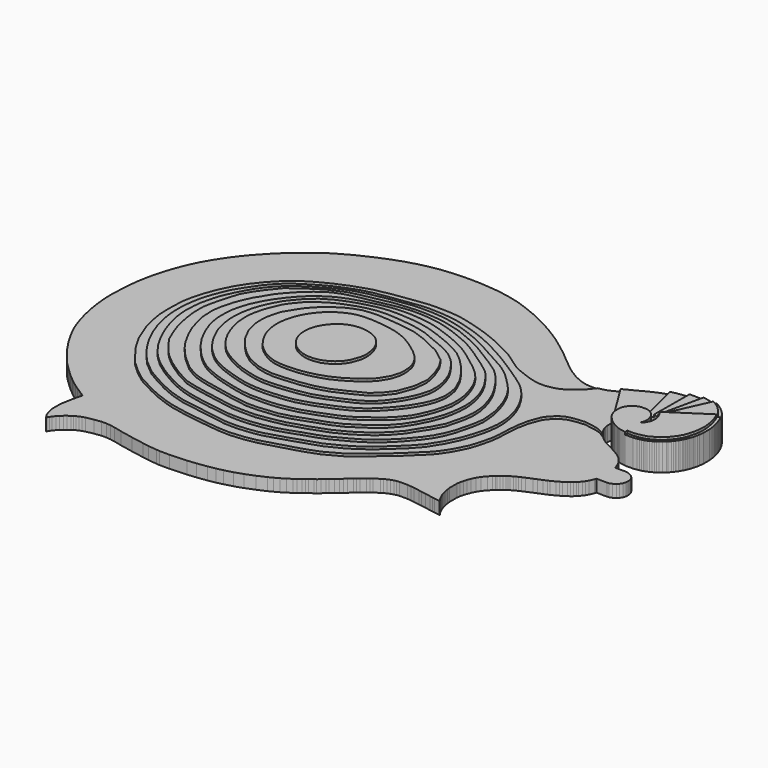
from build123d import *

# Parameters (mm, degrees)
F1_DEPTH  = 12
F2_DEPTH  = 11
F3_DEPTH  = 10
F4_DEPTH  = 9
F5_DEPTH  = 8
F6_DEPTH  = 7
F7_DEPTH  = 6
F8_DEPTH  = 16
F9_DEPTH  = 15
F10_DEPTH = 14
F11_DEPTH = 13
F12_DEPTH = 6
F13_DEPTH = 7
F14_DEPTH = 8
F15_DEPTH = 9
F16_DEPTH = 10
F17_DEPTH = 11
F18_DEPTH = 5


with BuildPart() as f1:
    # F0 (on Top) → F1 (new body)
    with BuildSketch(Plane.XY):
        Polygon((118.037871157, 25.3540883402), (102.8362065554, 15.362852253), (103.4810814802, 14.5440376551), (104.0835610836, 13.6208711236), (104.5890524983, 12.2988913208), (104.9133092165, 10.6635261327), (104.7770306468, 9.1832391918), (104.4950708747, 8.2950666547), (104.0034031764, 7.3146503921), (103.6714613438, 6.8094292656), (103.4511265296, 6.5506851914), (103.1008258023, 6.2215531917), (102.5383472443, 5.8092288673), (102.9038652778, 6.5668555908), (103.0799821019, 7.1051698178), (103.2660678029, 8.3977878094), (103.0932739377, 9.6272705123), (102.9005423188, 10.4081574827), (102.5110217551, 11.3447384652), (102.1528840065, 11.8935052305), (101.5746966004, 12.6112569124), (100.6889432971, 13.4109949539), (100.125901401, 13.7809263542), (99.7537374496, 13.9470724389), (99.1855189204, 14.1431251541), (98.261743784, 14.3292080611), (96.2148234248, 14.3292080611), (95.3331236025, 14.1279515674), (94.929825752, 13.9350700722), (94.2094346122, 13.5905353319), (93.6595828231, 13.231689472), (93.257419765, 12.8538291901), (92.5235550685, 12.1068896531), (92.1475663781, 11.5346284583), (91.7687490582, 10.7703544199), (91.5926322341, 10.268593207), (91.3999006152, 9.3082673848), (91.3999006152, 7.1284282021), (91.5801233458, 6.3727506401), (91.7958595391, 5.7682827865), (92.1503528953, 4.8411986791), (92.7119255066, 3.8077686913), (93.2867899537, 3.0235585291), (94.1274911165, 2.2061190102), (94.6957170963, 1.6013465356), (95.569640398, 0.8769488777), (96.3249058988, 0.3252295475), (96.9317836066, -0.0735029835), (97.5334867835, -0.4688357294), (98.8128110766, -1.0370564414), (99.1816520691, -1.2032024097), (99.7133255005, -1.4191925293), (100.2920271136, -1.6100962867), (101.059101522, -1.7980061239), (101.9629389048, -1.9774441607), (102.9066517949, -2.1502363961), (102.908693254, -0.9461662266), (104.2371541262, -1.030829153), (105.8742851019, -0.9717629873), (106.7681163549, -0.8665717323), (108.4452420473, -0.5530540366), (110.3363856673, 0), (112.0619401336, 0.9171339334), (113.7006878853, 1.8982925685), (115.3403148055, 3.3722929657), (116.4971739054, 4.6465592459), (117.7974045277, 6.501397118), (118.6752158388, 8.0567001438), (119.3536221981, 10.0181270391), (119.7435930371, 11.4179737866), (120.1347336173, 13.4776094928), (120.3220263124, 16.5463332087), (119.9393123388, 19.2720629275), (119.4058284163, 21.7033550143), (118.7055855989, 23.7527452409), align=None)
    extrude(amount=F1_DEPTH)


with BuildPart() as f1b:
    # F0 (on Top) → F1, piece 2 (new body)
    with BuildSketch(Plane.XY):
        Polygon((43.059155345, -18.4314288199), (43.059155345, -17.5313558429), (42.902559042, -15.3432423249), (42.4276590347, -12.6501116902), (41.5757112205, -10.4493321851), (40.020365268, -7.1345642209), (38.4353175759, -4.6706255525), (36.5965366364, -2.0937889349), (34.3441851437, 0.6145311636), (32.5511097908, 2.4446728639), (31.133595854, 3.9163869806), (29.2554348707, 5.4911249317), (27.8279818594, 6.6603217274), (25.8738175035, 7.800059393), (23.919634521, 8.9303422719), (20.2077943832, 10.6335915625), (15.1704987511, 12.6838255674), (12.0500344783, 13.7549508363), (9.9539672956, 14.4217368215), (7.0678894408, 15.0774177164), (3.485795809, 15.6938321888), (-0.4918280174, 16.006918624), (-3.040185431, 16.1812007427), (-6.7080380395, 16.1640755832), (-8.9749032632, 15.9702766687), (-11.7218578234, 15.5202383175), (-15.1372440159, 14.6717783064), (-17.8753435612, 13.9098102227), (-22.1570767462, 12.4261705205), (-25.1971576363, 11.077481322), (-29.3676964939, 8.6487792432), (-32.5607731938, 5.8629135601), (-33.6255170405, 4.716867581), (-35.5857908726, 2.3873208556), (-37.2510851825, 0.2279692002), (-39.0844345093, -3.0176998116), (-40.6988076866, -6.5281605348), (-41.7010299861, -9.5552252606), (-42.4500070512, -12.9693420604), (-42.6692888141, -14.6618969738), (-42.8908243775, -17.63317734), (-42.7832752466, -20.072389394), (-42.2973632812, -23.5900096595), (-41.3753129542, -27.1292198449), (-40.5848398805, -29.1735492647), (-39.3032543361, -31.7789278924), (-38.4896583855, -33.3960242569), (-36.8166342378, -36.0005907714), (-35.2769233286, -38.0995608866), (-33.7143093348, -39.8949608207), (-32.1399383247, -41.3643345237), (-30.3309373558, -42.9681055248), (-27.9739703983, -44.6044616401), (-24.5995428413, -46.4072935283), (-21.6266606003, -47.5926958025), (-18.0051922798, -48.8329418004), (-15.3112197295, -49.625467509), (-12.5499628484, -50.3166764975), (-9.8665812984, -50.7719777524), (-7.518351078, -51.0144010186), (-3.660001792, -51.107507199), (-0.4609905591, -50.9097017348), (1.6195356147, -50.7479719818), (4.158730153, -50.5178272724), (7.5596766546, -49.9598793685), (9.8199602216, -49.3368655443), (13.7588931248, -48.1257736683), (18.0006884038, -46.4081801474), (20.3957948834, -45.4363934696), (23.5745757818, -44.0133102238), (26.384525001, -42.4560904503), (29.3407179415, -40.4151715338), (31.7379795015, -38.2180400193), (33.7660089135, -36.1116230488), (35.1668149233, -34.5236249268), (36.9713753462, -32.2940051556), (38.2270030677, -30.5826552212), (39.7635288537, -28.1399991363), (40.784586221, -26.2605082244), (41.8287701905, -23.9537879825), (42.5147786736, -21.8051988631), (42.7293740213, -20.6131339073), (42.988628149, -19.4659456611), align=None)
        Polygon((38.576580584, -17.4344815314), (38.5574437678, -17.4484346062), (38.4194796867, -20.3703929465), (37.7189517021, -22.9599140584), (36.8902906775, -25.2610519528), (35.6621481478, -27.8303995728), (34.6747301519, -29.6506006271), (32.7814370394, -32.3015488684), (31.3950106502, -34.1225862503), (29.3429121375, -36.3193303347), (27.13201195, -38.06187585), (24.2294967175, -39.8058667779), (19.1714521497, -42.0623719692), (14.6992709488, -43.9433306456), (10.7068894431, -45.2618040144), (5.8373496868, -46.2077893317), (0.7289231871, -46.8601621687), (-2.7297076304, -47.1882410347), (-7.0656845346, -47.250777483), (-10.2039333433, -46.9097532332), (-13.5010341182, -46.1412630975), (-18.1004740298, -44.7605401278), (-21.2368406355, -43.3500185609), (-24.2931712419, -41.8056435883), (-26.8470719457, -40.2297824621), (-29.5722819865, -38.1220504642), (-32.2959497571, -35.137463361), (-33.8576920331, -32.847430557), (-35.5301275849, -29.9056153744), (-36.821834743, -26.6932006925), (-37.5780798495, -24.266589433), (-38.3105352521, -21.0305247456), (-38.5760738704, -17.4484346062), (-38.4340658784, -14.96030204), (-38.2297821343, -13.2736274973), (-37.3061597347, -9.5619428903), (-36.1824445426, -6.5468330868), (-34.8797030747, -3.486393718), (-33.4442593157, -1.2800322147), (-30.5974781513, 2.1433825605), (-28.5810474306, 4.0137115866), (-24.7513651848, 6.5993433818), (-22.0647975802, 8.051850833), (-19.6024682373, 9.091229178), (-15.282580629, 10.6965806335), (-11.948203668, 11.5579161793), (-8.5696056485, 12.1270604432), (-4.789091181, 12.2923450544), (-1.4342460781, 12.0745254681), (1.2719598599, 11.8778320029), (6.0577024706, 11.2807862461), (9.1210873798, 10.6801418588), (12.5194434077, 9.7654303536), (15.2910118923, 8.5796089843), (19.9626218528, 6.6782981157), (23.8517727703, 5.0226636231), (27.4716354907, 2.8718474787), (30.5537506938, 0.2027844457), (32.2725884616, -1.7946357839), (34.2138782144, -4.4885734096), (36.1319296062, -7.6771909371), (37.266407162, -10.5285858735), (38.0890294909, -13.3627839386), (38.4731926024, -15.7235115767), align=None, mode=Mode.SUBTRACT)
    extrude(amount=F1_DEPTH)

    # F0 (on Top) → F2, piece 2 (join)
    with BuildSketch(Plane.XY):
        Polygon((46.9649061561, -19.820921123), (46.9649061561, -17.5313558429), (46.9620004296, -16.0973109305), (46.6216802597, -12.9831163213), (46.0933409631, -10.8987120911), (45.3090779483, -8.4125790745), (44.3515963852, -5.9414184652), (43.2371608913, -3.6841758993), (41.5528938174, -1.113338978), (39.9568453431, 0.7494483725), (37.9806607962, 2.678884659), (35.903442651, 4.3945279904), (32.7515788376, 6.7609921098), (30.4898880422, 8.5155731067), (26.1934623122, 11.4335659891), (23.6024521291, 12.871962972), (20.8515319973, 14.1362315044), (18.725162372, 15.0809623301), (15.7878063619, 16.2111781538), (13.3554367349, 17.1017926186), (11.0558578745, 17.8723614663), (9.5670297742, 18.3237846941), (7.1474183351, 18.9069472253), (5.0731659867, 19.2368254066), (3.1982769724, 19.4869115949), (1.083960291, 19.7231266648), (-1.8417660613, 19.9041739106), (-5.0983610563, 19.8868848383), (-6.9992956705, 19.7640750557), (-9.3089621514, 19.5207744837), (-12.3783918098, 18.9579259604), (-16.63486287, 17.9474465549), (-19.7523571551, 17.0347392559), (-23.1864396483, 15.9782916307), (-25.4973098636, 15.0513732806), (-27.8242472559, 13.9813376591), (-31.2603451312, 11.7802238092), (-33.7784551084, 9.9307820201), (-36.6303361952, 7.1585532278), (-39.4199341536, 3.8300235756), (-41.5445566177, 0.8844275144), (-43.1148074567, -1.6148544382), (-44.6226559579, -4.6068299562), (-45.6864908338, -6.9460715167), (-46.8957275152, -11.0185155645), (-47.3741739988, -13.2611459121), (-47.5535579026, -16.3298584521), (-47.5438944995, -19.8274180293), (-46.9183623791, -23.8801315427), (-46.4623346925, -25.3894980997), (-44.9195094407, -29.4879861176), (-42.5710193813, -34.1412238777), (-39.8102477193, -38.2053554058), (-36.6535000503, -41.9507063925), (-34.4272814691, -44.1876836121), (-32.105602324, -46.106506139), (-30.2258692682, -47.5016087294), (-27.8242137283, -48.9115193486), (-23.0827387422, -50.9206689894), (-19.684093073, -52.0264320076), (-14.0085108578, -53.5089969635), (-10.1348320022, -54.3117001653), (-6.7350403406, -54.7509230673), (-3.5241844598, -54.7509230673), (0.3034151741, -54.7509230673), (4.3689650483, -54.3767698109), (8.1344619393, -53.7329725921), (11.8687273934, -52.8666712344), (17.0755460858, -51.0911010206), (21.9029858708, -49.1891354322), (23.8180737942, -48.4697185457), (25.7650725543, -47.5912503898), (28.3299610019, -46.1232662201), (30.8636054397, -44.4327779114), (36.1377485096, -40.3518415987), (38.5933183134, -38.0891822278), (40.5904091895, -35.7161797583), (41.8427325785, -34.1237559915), (43.080329895, -31.9113321602), (44.445939362, -28.8560595363), (45.4152673483, -26.2944418937), (46.1791716516, -23.6219670624), (46.5301908553, -21.8883417547), align=None)
        Polygon((42.902559042, -15.3432423249), (43.059155345, -17.5313558429), (43.059155345, -18.4314288199), (42.988628149, -19.4659456611), (42.7293740213, -20.6131339073), (42.5147786736, -21.8051988631), (41.8287701905, -23.9537879825), (40.784586221, -26.2605082244), (39.7635288537, -28.1399991363), (38.2270030677, -30.5826552212), (36.9713753462, -32.2940051556), (35.1668149233, -34.5236249268), (33.7660089135, -36.1116230488), (31.7379795015, -38.2180400193), (29.3407179415, -40.4151715338), (26.384525001, -42.4560904503), (23.5745757818, -44.0133102238), (20.3957948834, -45.4363934696), (18.0006884038, -46.4081801474), (13.7588931248, -48.1257736683), (9.8199602216, -49.3368655443), (7.5596766546, -49.9598793685), (4.158730153, -50.5178272724), (1.6195356147, -50.7479719818), (-0.4609905591, -50.9097017348), (-3.660001792, -51.107507199), (-7.518351078, -51.0144010186), (-9.8665812984, -50.7719777524), (-12.5499628484, -50.3166764975), (-15.3112197295, -49.625467509), (-18.0051922798, -48.8329418004), (-21.6266606003, -47.5926958025), (-24.5995428413, -46.4072935283), (-27.9739703983, -44.6044616401), (-30.3309373558, -42.9681055248), (-32.1399383247, -41.3643345237), (-33.7143093348, -39.8949608207), (-35.2769233286, -38.0995608866), (-36.8166342378, -36.0005907714), (-38.4896583855, -33.3960242569), (-39.3032543361, -31.7789278924), (-40.5848398805, -29.1735492647), (-41.3753129542, -27.1292198449), (-42.2973632812, -23.5900096595), (-42.7832752466, -20.072389394), (-42.8908243775, -17.63317734), (-42.6692888141, -14.6618969738), (-42.4500070512, -12.9693420604), (-41.7010299861, -9.5552252606), (-40.6988076866, -6.5281605348), (-39.0844345093, -3.0176998116), (-37.2510851825, 0.2279692002), (-35.5857908726, 2.3873208556), (-33.6255170405, 4.716867581), (-32.5607731938, 5.8629135601), (-29.3676964939, 8.6487792432), (-25.1971576363, 11.077481322), (-22.1570767462, 12.4261705205), (-17.8753435612, 13.9098102227), (-15.1372440159, 14.6717783064), (-11.7218578234, 15.5202383175), (-8.9749032632, 15.9702766687), (-6.7080380395, 16.1640755832), (-3.040185431, 16.1812007427), (-0.4918280174, 16.006918624), (3.485795809, 15.6938321888), (7.0678894408, 15.0774177164), (9.9539672956, 14.4217368215), (12.0500344783, 13.7549508363), (15.1704987511, 12.6838255674), (20.2077943832, 10.6335915625), (23.919634521, 8.9303422719), (25.8738175035, 7.800059393), (27.8279818594, 6.6603217274), (29.2554348707, 5.4911249317), (31.133595854, 3.9163869806), (32.5511097908, 2.4446728639), (34.3441851437, 0.6145311636), (36.5965366364, -2.0937889349), (38.4353175759, -4.6706255525), (40.020365268, -7.1345642209), (41.5757112205, -10.4493321851), (42.4276590347, -12.6501116902), align=None, mode=Mode.SUBTRACT)
    extrude(amount=F2_DEPTH)

    # F0 (on Top) → F3, piece 2 (join)
    with BuildSketch(Plane.XY):
        Polygon((44.5869043469, -34.9130816758), (45.709233731, -32.684892416), (45.7351990044, -32.6676554978), (47.1320189536, -29.8666413873), (48.5685840249, -25.8555412292), (49.3081398308, -22.4508922547), (49.7652962804, -19.1980861127), (49.8640015721, -16.5510196239), (49.7927255929, -14.301341027), (49.2344647646, -10.8805019408), (48.3185909688, -7.5927539729), (47.1762754023, -4.7213993967), (45.5642230809, -1.5674367314), (43.2566255331, 1.8119369633), (41.7930185795, 3.8129263557), (40.1970483363, 5.4166102782), (39.0514396131, 6.4162411727), (35.4071743786, 9.1121988371), (32.814539969, 10.8461417258), (29.6772606671, 13.0516011268), (25.6752837449, 15.5577473342), (22.5935354829, 17.2528568655), (18.9472381026, 18.7955386937), (14.7744482383, 20.4316526651), (11.1883048909, 21.6134019169), (8.0442121252, 22.4216338247), (5.7501969859, 22.8327736259), (2.9858469497, 23.1862105429), (0.0520141293, 23.4258603305), (-3.5781676415, 23.4371777624), (-5.8168186806, 23.2434384525), (-9.4479322433, 22.7253846824), (-12.2514972463, 22.1712477505), (-16.2028688937, 21.3689319789), (-20.5868408084, 20.5657333136), (-23.3152024448, 19.9928451329), (-26.3259708881, 19.2681197077), (-28.320863843, 18.6400488019), (-30.9559460729, 17.6325142384), (-33.1022106111, 16.4936613292), (-36.172144115, 14.2184859142), (-39.5065657794, 11.2810665742), (-43.313447386, 7.0759374648), (-45.0667105615, 4.8035373911), (-47.104138881, 1.3772920938), (-48.7451814115, -1.2540896423), (-50.3317266703, -4.9819247797), (-51.2219112371, -7.1146843555), (-52.6982955635, -12.8579484299), (-53.0393570662, -16.0063225776), (-52.7581460774, -21.4467104524), (-50.7801510394, -28.7046935409), (-48.9086955786, -32.9501219094), (-46.2554618716, -37.8234572709), (-43.9126454294, -41.1460883915), (-40.162332356, -45.4325601459), (-34.8023362458, -50.187818706), (-31.8082310259, -52.0251840353), (-29.6627748758, -53.0998967588), (-26.8013365567, -54.0606975555), (-23.8054133952, -54.863832891), (-12.4017419294, -57.2007410228), (-8.801558055, -57.8227490187), (-5.1116631366, -58.3906285465), (-0.8171134396, -58.3906285465), (3.3441430423, -57.9547323287), (6.8565160036, -57.632625103), (11.757383123, -56.3633181155), (18.2258486748, -54.056506604), (23.5079247504, -52.2468052804), (27.9179960489, -50.2365715802), (33.4268510342, -46.6726869345), (38.4439155459, -42.9299734533), (42.0523956418, -38.8304702938), align=None)
        Polygon((46.9620004296, -16.0973109305), (46.9649061561, -17.5313558429), (46.9649061561, -19.820921123), (46.5301908553, -21.8883417547), (46.1791716516, -23.6219670624), (45.4152673483, -26.2944418937), (44.445939362, -28.8560595363), (43.080329895, -31.9113321602), (41.8427325785, -34.1237559915), (40.5904091895, -35.7161797583), (38.5933183134, -38.0891822278), (36.1377485096, -40.3518415987), (30.8636054397, -44.4327779114), (28.3299610019, -46.1232662201), (25.7650725543, -47.5912503898), (23.8180737942, -48.4697185457), (21.9029858708, -49.1891354322), (17.0755460858, -51.0911010206), (11.8687273934, -52.8666712344), (8.1344619393, -53.7329725921), (4.3689650483, -54.3767698109), (0.3034151741, -54.7509230673), (-3.5241844598, -54.7509230673), (-6.7350403406, -54.7509230673), (-10.1348320022, -54.3117001653), (-14.0085108578, -53.5089969635), (-19.684093073, -52.0264320076), (-23.0827387422, -50.9206689894), (-27.8242137283, -48.9115193486), (-30.2258692682, -47.5016087294), (-32.105602324, -46.106506139), (-34.4272814691, -44.1876836121), (-36.6535000503, -41.9507063925), (-39.8102477193, -38.2053554058), (-42.5710193813, -34.1412238777), (-44.9195094407, -29.4879861176), (-46.4623346925, -25.3894980997), (-46.9183623791, -23.8801315427), (-47.5438944995, -19.8274180293), (-47.5535579026, -16.3298584521), (-47.3741739988, -13.2611459121), (-46.8957275152, -11.0185155645), (-45.6864908338, -6.9460715167), (-44.6226559579, -4.6068299562), (-43.1148074567, -1.6148544382), (-41.5445566177, 0.8844275144), (-39.4199341536, 3.8300235756), (-36.6303361952, 7.1585532278), (-33.7784551084, 9.9307820201), (-31.2603451312, 11.7802238092), (-27.8242472559, 13.9813376591), (-25.4973098636, 15.0513732806), (-23.1864396483, 15.9782916307), (-19.7523571551, 17.0347392559), (-16.63486287, 17.9474465549), (-12.3783918098, 18.9579259604), (-9.3089621514, 19.5207744837), (-6.9992956705, 19.7640750557), (-5.0983610563, 19.8868848383), (-1.8417660613, 19.9041739106), (1.083960291, 19.7231266648), (3.1982769724, 19.4869115949), (5.0731659867, 19.2368254066), (7.1474183351, 18.9069472253), (9.5670297742, 18.3237846941), (11.0558578745, 17.8723614663), (13.3554367349, 17.1017926186), (15.7878063619, 16.2111781538), (18.725162372, 15.0809623301), (20.8515319973, 14.1362315044), (23.6024521291, 12.871962972), (26.1934623122, 11.4335659891), (30.4898880422, 8.5155731067), (32.7515788376, 6.7609921098), (35.903442651, 4.3945279904), (37.9806607962, 2.678884659), (39.9568453431, 0.7494483725), (41.5528938174, -1.113338978), (43.2371608913, -3.6841758993), (44.3515963852, -5.9414184652), (45.3090779483, -8.4125790745), (46.0933409631, -10.8987120911), (46.6216802597, -12.9831163213), align=None, mode=Mode.SUBTRACT)
    extrude(amount=F3_DEPTH)

    # F0 (on Top) → F4 (join)
    with BuildSketch(Plane.XY):
        Polygon((53.4976534545, -20.8242163062), (53.8227409124, -17.481373623), (53.7689168697, -16.1077379619), (53.596008569, -13.3690275252), (52.9684312642, -10.4956282303), (52.0563200116, -7.4899541214), (50.6704859436, -4.058863502), (48.9678196609, -0.9146001539), (46.3491752744, 3.0226481613), (44.6449965239, 5.3084110841), (42.4033813179, 7.7838273719), (40.3188727796, 9.6554430202), (38.4232103825, 10.9869204462), (36.5590713918, 12.254871428), (30.5868908763, 15.9625392407), (26.3525284827, 18.5291841626), (22.7811858058, 20.3658975661), (19.209228456, 21.852850914), (15.130232775, 23.5529562425), (11.1710579004, 24.5707161181), (7.8591220081, 25.4220943898), (4.1905259714, 25.9231589735), (-0.5221402389, 26.3266582042), (-3.7775287285, 26.3398705633), (-7.167742122, 26.1258296669), (-13.1566778702, 25.5151093117), (-19.2119580103, 24.2908696707), (-25.2242386341, 23.0753235519), (-29.1180610657, 22.0779180527), (-35.0726880133, 19.4124355912), (-41.1626771092, 15.5660808086), (-46.271879226, 11.7057748139), (-49.9556176364, 7.1521895006), (-52.5690577924, 3.4035053104), (-54.4922798439, 0), (-55.8674678143, -4.2537574426), (-57.5681366026, -10.8695076779), (-58.1104531884, -14.0523137525), (-58.1104531884, -16.7261101305), (-58.0355450511, -19.5066314191), (-57.4523048098, -23.5256252818), (-56.4816407859, -28.3266808838), (-54.9996346235, -32.6550267637), (-52.8804883361, -37.7039462328), (-50.2271652222, -41.5218323469), (-46.271879226, -46.1658537388), (-42.3144288361, -49.579963088), (-39.4451022148, -51.5792667866), (-36.0175892711, -53.8180321455), (-30.4604840677, -56.7577148281), (-25.6507750601, -57.9941160977), (-20.7314211875, -58.9731112123), (-14.3759222701, -60.1095221937), (-8.8447583839, -61.087243259), (-4.4028488919, -61.2546615303), (0.5980937276, -61.2546615303), (6.2289447031, -60.4221399338), (11.4809926599, -59.3602955341), (18.7735296786, -57.072378695), (25.906983763, -54.490685463), (31.4181819558, -51.6984947026), (34.8535552621, -49.4721159339), (37.9962734878, -47.2730882466), (41.4599813521, -44.0573655069), (44.6585379541, -40.3609350324), (46.9261221588, -36.6397090256), (49.1932332516, -33.1858582795), (51.6020112706, -28.5715754719), (52.7202636003, -24.2214761674), align=None)
        Polygon((45.7351990044, -32.6676554978), (45.709233731, -32.684892416), (44.5869043469, -34.9130816758), (42.0523956418, -38.8304702938), (38.4439155459, -42.9299734533), (33.4268510342, -46.6726869345), (27.9179960489, -50.2365715802), (23.5079247504, -52.2468052804), (18.2258486748, -54.056506604), (11.757383123, -56.3633181155), (6.8565160036, -57.632625103), (3.3441430423, -57.9547323287), (-0.8171134396, -58.3906285465), (-5.1116631366, -58.3906285465), (-8.801558055, -57.8227490187), (-12.4017419294, -57.2007410228), (-23.8054133952, -54.863832891), (-26.8013365567, -54.0606975555), (-29.6627748758, -53.0998967588), (-31.8082310259, -52.0251840353), (-34.8023362458, -50.187818706), (-40.162332356, -45.4325601459), (-43.9126454294, -41.1460883915), (-46.2554618716, -37.8234572709), (-48.9086955786, -32.9501219094), (-50.7801510394, -28.7046935409), (-52.7581460774, -21.4467104524), (-53.0393570662, -16.0063225776), (-52.6982955635, -12.8579484299), (-51.2219112371, -7.1146843555), (-50.3317266703, -4.9819247797), (-48.7451814115, -1.2540896423), (-47.104138881, 1.3772920938), (-45.0667105615, 4.8035373911), (-43.313447386, 7.0759374648), (-39.5065657794, 11.2810665742), (-36.172144115, 14.2184859142), (-33.1022106111, 16.4936613292), (-30.9559460729, 17.6325142384), (-28.320863843, 18.6400488019), (-26.3259708881, 19.2681197077), (-23.3152024448, 19.9928451329), (-20.5868408084, 20.5657333136), (-16.2028688937, 21.3689319789), (-12.2514972463, 22.1712477505), (-9.4479322433, 22.7253846824), (-5.8168186806, 23.2434384525), (-3.5781676415, 23.4371777624), (0.0520141293, 23.4258603305), (2.9858469497, 23.1862105429), (5.7501969859, 22.8327736259), (8.0442121252, 22.4216338247), (11.1883048909, 21.6134019169), (14.7744482383, 20.4316526651), (18.9472381026, 18.7955386937), (22.5935354829, 17.2528568655), (25.6752837449, 15.5577473342), (29.6772606671, 13.0516011268), (32.814539969, 10.8461417258), (35.4071743786, 9.1121988371), (39.0514396131, 6.4162411727), (40.1970483363, 5.4166102782), (41.7930185795, 3.8129263557), (43.2566255331, 1.8119369633), (45.5642230809, -1.5674367314), (47.1762754023, -4.7213993967), (48.3185909688, -7.5927539729), (49.2344647646, -10.8805019408), (49.7927255929, -14.301341027), (49.8640015721, -16.5510196239), (49.7652962804, -19.1980861127), (49.3081398308, -22.4508922547), (48.5685840249, -25.8555412292), (47.1320189536, -29.8666413873), align=None, mode=Mode.SUBTRACT)
    extrude(amount=F4_DEPTH)

    # F0 (on Top) → F5, piece 2 (join)
    with BuildSketch(Plane.XY):
        Polygon((57.7011555433, -14.9035872892), (57.2556294501, -11.1078219488), (56.7832998931, -9.1371238232), (56.0915581882, -6.7538553849), (55.210467428, -4.1166162118), (53.8555122912, -1.1147102341), (53.0201606452, 0.5528439651), (51.4584705234, 2.9183875304), (50.5747757852, 4.0771006607), (48.8225854933, 6.0448022559), (45.85429281, 9.0274335817), (43.454118073, 11.2799424678), (41.2743464112, 12.9446852952), (39.4576303661, 14.1968326643), (35.791773349, 16.2559244782), (30.3244907409, 19.2651338875), (26.5322551131, 21.4034561068), (22.9135211557, 23.2718642801), (20.2741641551, 24.4269073009), (16.9391781092, 25.7553756237), (13.6039694771, 26.9566588104), (9.9363001063, 27.9823690653), (6.3315662555, 28.8174450397), (2.457439201, 29.3657816947), (-0.9426044999, 29.6129867338), (-5.3699262171, 29.6129867338), (-8.6458129808, 29.4061638415), (-13.6451404542, 28.6962036043), (-17.2782458299, 28.1820992578), (-19.6730587631, 27.6979226619), (-22.4491620502, 27.1731853963), (-25.1791644841, 26.6212411225), (-28.2491259277, 25.7563274354), (-30.9554152191, 24.8285792768), (-34.0895093977, 23.4706904739), (-37.3982638121, 21.730883047), (-41.3248203695, 19.4492451847), (-43.4149801731, 18.1094370782), (-45.7113198936, 16.4512339979), (-47.9605197906, 14.6182533354), (-49.0378215909, 13.6144217104), (-50.9709902108, 11.6072213277), (-52.9366061091, 9.1389082372), (-54.3954409659, 7.0373108611), (-56.3469193876, 3.6151239183), (-57.7592775226, 0.9571905248), (-59.6859327434, -3.5658766784), (-60.4921020567, -6.0595348477), (-61.6392754018, -10.8154667541), (-61.9610659778, -13.9162680134), (-62.1365492395, -17.5589057148), (-61.9720630348, -20.1642177999), (-61.6450347006, -23.0728853494), (-60.6629960239, -27.2758472711), (-59.1497644782, -31.7131206393), (-57.8800924122, -34.7344689071), (-56.2146045268, -38.2026098669), (-54.0000461042, -41.9412106276), (-52.0363338292, -44.6242019534), (-49.7137755156, -47.4534966052), (-46.3277362287, -50.5880489945), (-42.6084622741, -53.3074773848), (-40.1241406798, -54.9065247178), (-37.9052124918, -56.1585389078), (-35.0485518575, -57.7969141304), (-31.6862948239, -59.3272745609), (-29.0414243937, -60.3912398219), (-25.704825297, -61.3869167864), (-21.5035490692, -62.2872039676), (-16.5573693812, -63.1729438901), (-10.8403386548, -63.9831200242), (-7.3708849959, -64.4768774509), (-5.3493888117, -64.5528659225), (-1.6266150137, -64.5794949829), (0.6891145022, -64.4332915545), (5.8507905342, -63.7540742755), (9.8954793066, -62.9435032606), (14.63291049, -61.4897869527), (18.093187362, -60.2258965373), (23.2566520572, -58.5306547582), (27.1163601428, -57.0253022015), (29.4594187289, -55.7637475431), (33.240173012, -53.7772737443), (36.5153253078, -51.8988147378), (39.5249500871, -49.7535392642), (42.7750572562, -46.9928048551), (45.8661280572, -43.9115576446), (50.1310154796, -38.9027483761), (52.344456315, -35.7163846493), (54.0525764227, -32.4776172638), (55.4688982666, -28.7849083543), (56.4866773784, -24.8256586492), (57.2368092835, -21.8027774245), (57.8692729799, -17.5664147896), align=None)
        Polygon((53.7689168697, -16.1077379619), (53.8227409124, -17.481373623), (53.4976534545, -20.8242163062), (52.7202636003, -24.2214761674), (51.6020112706, -28.5715754719), (49.1932332516, -33.1858582795), (46.9261221588, -36.6397090256), (44.6585379541, -40.3609350324), (41.4599813521, -44.0573655069), (37.9962734878, -47.2730882466), (34.8535552621, -49.4721159339), (31.4181819558, -51.6984947026), (25.906983763, -54.490685463), (18.7735296786, -57.072378695), (11.4809926599, -59.3602955341), (6.2289447031, -60.4221399338), (0.5980937276, -61.2546615303), (-4.4028488919, -61.2546615303), (-8.8447583839, -61.087243259), (-14.3759222701, -60.1095221937), (-20.7314211875, -58.9731112123), (-25.6507750601, -57.9941160977), (-30.4604840677, -56.7577148281), (-36.0175892711, -53.8180321455), (-39.4451022148, -51.5792667866), (-42.3144288361, -49.579963088), (-46.271879226, -46.1658537388), (-50.2271652222, -41.5218323469), (-52.8804883361, -37.7039462328), (-54.9996346235, -32.6550267637), (-56.4816407859, -28.3266808838), (-57.4523048098, -23.5256252818), (-58.0355450511, -19.5066314191), (-58.1104531884, -16.7261101305), (-58.1104531884, -14.0523137525), (-57.5681366026, -10.8695076779), (-55.8674678143, -4.2537574426), (-54.4922798439, 0), (-52.5690577924, 3.4035053104), (-49.9556176364, 7.1521895006), (-46.271879226, 11.7057748139), (-41.1626771092, 15.5660808086), (-35.0726880133, 19.4124355912), (-29.1180610657, 22.0779180527), (-25.2242386341, 23.0753235519), (-19.2119580103, 24.2908696707), (-13.1566778702, 25.5151093117), (-7.167742122, 26.1258296669), (-3.7775287285, 26.3398705633), (-0.5221402389, 26.3266582042), (4.1905259714, 25.9231589735), (7.8591220081, 25.4220943898), (11.1710579004, 24.5707161181), (15.130232775, 23.5529562425), (19.209228456, 21.852850914), (22.7811858058, 20.3658975661), (26.3525284827, 18.5291841626), (30.5868908763, 15.9625392407), (36.5590713918, 12.254871428), (38.4232103825, 10.9869204462), (40.3188727796, 9.6554430202), (42.4033813179, 7.7838273719), (44.6449965239, 5.3084110841), (46.3491752744, 3.0226481613), (48.9678196609, -0.9146001539), (50.6704859436, -4.058863502), (52.0563200116, -7.4899541214), (52.9684312642, -10.4956282303), (53.596008569, -13.3690275252), align=None, mode=Mode.SUBTRACT)
    extrude(amount=F5_DEPTH)

    # F0 (on Top) → F6 (join)
    with BuildSketch(Plane.XY):
        Polygon((62.2659102082, -12.919511646), (62.0128065348, -10.4956282303), (61.3787025213, -7.3592509143), (60.4352615774, -4.1975039057), (58.7968118489, -0.4966377585), (56.6994249821, 3.0283040833), (55.1216416061, 5.2348412573), (53.0379153788, 7.5516202487), (51.5220835805, 9.0110758319), (50.1163974404, 10.1527804509), (47.288864851, 12.2295189649), (42.7864082158, 15.2407586575), (37.7782024443, 18.4735134244), (33.1172421575, 21.2936345488), (28.7244059145, 23.6850641668), (25.7062315941, 25.2844598144), (20.5224212259, 27.5947451591), (16.7580679024, 29.0099394538), (14.6042127162, 29.7062546015), (10.704212822, 30.8617763221), (7.7262255363, 31.5774604678), (3.9499443956, 32.1310535073), (1.2903637253, 32.3928669095), (-4.4077960774, 32.6058194041), (-7.55826151, 32.4069149792), (-18.5202583671, 30.9134498239), (-24.4006179273, 29.965352267), (-28.3657871187, 28.9945211262), (-33.1567935646, 27.3267962039), (-37.9220023751, 25.2045895904), (-41.4898097515, 23.2987813652), (-46.4694239199, 20.2670581639), (-50.0117614865, 17.7196115255), (-53.0762784183, 14.611678198), (-55.3953684866, 11.8528883904), (-58.9424557984, 6.6049606539), (-61.1835792661, 2.8035794385), (-63.3800654021, -2.6882183855), (-64.6582618356, -6.6419597715), (-65.4104650021, -10.8412886038), (-65.8503249288, -14.4518259913), (-65.8503249288, -18.9435966313), (-65.5894502997, -21.8574162573), (-65.1161447167, -24.984691292), (-64.0596970916, -29.2871817946), (-62.2595660388, -34.2298187315), (-59.8742738366, -39.1979701817), (-57.0892654359, -43.7642261386), (-54.5680522919, -47.0744036138), (-51.3295680285, -50.9178005159), (-45.7107424736, -55.6248798966), (-41.1285832524, -58.2861788571), (-36.3247655332, -60.8198344707), (-31.8362191319, -62.7500265837), (-28.6114457995, -63.7925565243), (-25.8923657238, -64.5817816257), (-12.3255038634, -66.7791515589), (-6.4749824814, -67.7208155394), (-1.9199246308, -67.8066760302), (2.161302371, -67.5119832158), (6.2429797836, -66.9629126787), (8.4899095818, -66.4176791906), (15.8011130989, -64.2084628344), (27.1957702935, -60.4326948524), (32.9580493271, -57.5907900929), (36.9480699301, -55.1977343857), (40.9074053168, -52.2642098367), (43.5686483979, -49.96933043), (49.3354052305, -44.583722949), (52.9487356544, -40.5380539596), (56.5017089248, -34.8391085863), (58.78771469, -30.064901337), (60.3774823248, -25.4511535168), (61.5237914026, -21.1880709976), (62.0032176375, -18.3890033513), (62.260761857, -15.8447716385), align=None)
        Polygon((56.7832998931, -9.1371238232), (57.2556294501, -11.1078219488), (57.7011555433, -14.9035872892), (57.8692729799, -17.5664147896), (57.2368092835, -21.8027774245), (56.4866773784, -24.8256586492), (55.4688982666, -28.7849083543), (54.0525764227, -32.4776172638), (52.344456315, -35.7163846493), (50.1310154796, -38.9027483761), (45.8661280572, -43.9115576446), (42.7750572562, -46.9928048551), (39.5249500871, -49.7535392642), (36.5153253078, -51.8988147378), (33.240173012, -53.7772737443), (29.4594187289, -55.7637475431), (27.1163601428, -57.0253022015), (23.2566520572, -58.5306547582), (18.093187362, -60.2258965373), (14.63291049, -61.4897869527), (9.8954793066, -62.9435032606), (5.8507905342, -63.7540742755), (0.6891145022, -64.4332915545), (-1.6266150137, -64.5794949829), (-5.3493888117, -64.5528659225), (-7.3708849959, -64.4768774509), (-10.8403386548, -63.9831200242), (-16.5573693812, -63.1729438901), (-21.5035490692, -62.2872039676), (-25.704825297, -61.3869167864), (-29.0414243937, -60.3912398219), (-31.6862948239, -59.3272745609), (-35.0485518575, -57.7969141304), (-37.9052124918, -56.1585389078), (-40.1241406798, -54.9065247178), (-42.6084622741, -53.3074773848), (-46.3277362287, -50.5880489945), (-49.7137755156, -47.4534966052), (-52.0363338292, -44.6242019534), (-54.0000461042, -41.9412106276), (-56.2146045268, -38.2026098669), (-57.8800924122, -34.7344689071), (-59.1497644782, -31.7131206393), (-60.6629960239, -27.2758472711), (-61.6450347006, -23.0728853494), (-61.9720630348, -20.1642177999), (-62.1365492395, -17.5589057148), (-61.9610659778, -13.9162680134), (-61.6392754018, -10.8154667541), (-60.4921020567, -6.0595348477), (-59.6859327434, -3.5658766784), (-57.7592775226, 0.9571905248), (-56.3469193876, 3.6151239183), (-54.3954409659, 7.0373108611), (-52.9366061091, 9.1389082372), (-50.9709902108, 11.6072213277), (-49.0378215909, 13.6144217104), (-47.9605197906, 14.6182533354), (-45.7113198936, 16.4512339979), (-43.4149801731, 18.1094370782), (-41.3248203695, 19.4492451847), (-37.3982638121, 21.730883047), (-34.0895093977, 23.4706904739), (-30.9554152191, 24.8285792768), (-28.2491259277, 25.7563274354), (-25.1791644841, 26.6212411225), (-22.4491620502, 27.1731853963), (-19.6730587631, 27.6979226619), (-17.2782458299, 28.1820992578), (-13.6451404542, 28.6962036043), (-8.6458129808, 29.4061638415), (-5.3699262171, 29.6129867338), (-0.9426044999, 29.6129867338), (2.457439201, 29.3657816947), (6.3315662555, 28.8174450397), (9.9363001063, 27.9823690653), (13.6039694771, 26.9566588104), (16.9391781092, 25.7553756237), (20.2741641551, 24.4269073009), (22.9135211557, 23.2718642801), (26.5322551131, 21.4034561068), (30.3244907409, 19.2651338875), (35.791773349, 16.2559244782), (39.4576303661, 14.1968326643), (41.2743464112, 12.9446852952), (43.454118073, 11.2799424678), (45.85429281, 9.0274335817), (48.8225854933, 6.0448022559), (50.5747757852, 4.0771006607), (51.4584705234, 2.9183875304), (53.0201606452, 0.5528439651), (53.8555122912, -1.1147102341), (55.210467428, -4.1166162118), (56.0915581882, -6.7538553849), align=None, mode=Mode.SUBTRACT)
    extrude(amount=F6_DEPTH)

    # F0 (on Top) → F7 (join)
    with BuildSketch(Plane.XY):
        Polygon((88.6424705386, 9.3967169523), (77.4692744017, 27.3676645011), (75.9997218847, 26.7088897526), (73.6500956581, 25.5534786533), (70.8051025867, 24.8641371727), (70.3159928804, 24.8075255182), (68.3903247118, 22.3890021443), (66.7697489262, 20.7029692829), (64.8483708501, 19.0919302404), (63.3417516947, 18.0300362408), (61.4025220275, 16.967240721), (59.3321882188, 16.2255745381), (56.3782453537, 15.7278385013), (54.5160472393, 15.6861338764), (52.8259277344, 15.833940357), (50.4111051559, 16.3684915751), (47.1920520067, 17.4859277904), (44.8673330247, 18.380401656), (42.9896637797, 19.0959405154), (40.9337617457, 20.2158074826), (37.7613417804, 22.4125385284), (33.9634120464, 25.0576287508), (30.2983354777, 26.9385650754), (24.9346978962, 29.6253506094), (18.9889334142, 31.9961495697), (13.4447673336, 33.78322348), (9.2862462625, 34.8986983299), (5.1274085417, 35.8343012631), (0.6096527213, 36.1845940351), (-3.7296339869, 36.2654626369), (-6.9507444277, 36.2137593329), (-12.7677610144, 35.48213467), (-20.5090809613, 34.3867540359), (-27.3561477661, 33.023443073), (-34.2047959566, 30.7608004659), (-39.6667681634, 28.4111201763), (-44.8160618544, 25.7922913879), (-49.1601750255, 23.1301821768), (-53.4164011478, 19.5689257234), (-56.957077235, 15.8742628992), (-60.2301247418, 11.7305023596), (-62.9664957523, 7.497922983), (-65.4808357358, 2.3215094116), (-67.3176944256, -2.5615892373), (-68.3408276406, -6.2728059455), (-69.0556520852, -9.8359373647), (-69.1953599453, -11.3946693018), (-69.3785399199, -15.3844263405), (-69.3785399199, -19.2977990955), (-69.2147761583, -22.4358737469), (-68.490414488, -26.4581795747), (-67.3678815365, -31.0910046101), (-64.2780438066, -38.8738662004), (-61.1839145422, -44.2178547382), (-57.267686539, -49.4970759001), (-54.9507598676, -52.4328832321), (-50.3715239465, -56.5976724029), (-46.3329255581, -59.6709251404), (-39.8685485125, -63.0983263254), (-35.7106773342, -65.0627390351), (-30.733935535, -66.9171735644), (-27.7962588841, -67.8310851114), (-20.8630915731, -69.2219957709), (-11.3479318097, -70.5633535981), (-6.1763790436, -71.1386278272), (-1.5496322885, -71.3369250298), (3.7930996623, -70.8342045546), (8.6098033935, -69.9733570218), (22.9309424758, -65.8596977592), (29.0855076164, -63.6348202825), (35.5588686626, -60.1097050092), (41.8343506753, -55.1571212709), (48.7333716388, -49.3617232165), (56.5668642521, -41.7407862842), (58.0184161663, -39.9038530886), (59.0178407729, -38.4648963809), (60.3757463396, -36.4012904465), (61.5835040808, -34.1489315033), (63.1314665079, -30.9694670141), (64.3608868122, -27.0911473781), (65.5357912183, -22.1352875233), (65.8232197165, -19.128613174), (65.9816306986, -14.7936397301), (66.3495704762, -10.6885057619), (67.2079631219, -6.409740774), (68.0863347919, -4.0524566875), (68.8818097115, -1.9176424248), (69.8404767737, -0.4966377585), (70.6509101132, 0.3944434722), (71.7846378684, 1.4974084136), (72.8580728173, 2.344558714), (74.7373939507, 3.346915398), (76.6413286328, 3.8082385436), (78.9554864168, 4.1533852927), (81.5891325474, 4.3479516171), (85.970453918, 3.6386775319), (88.0384594202, 3.056909889), (89.8049771786, 2.172014676), (91.5926322341, 0.966749154), (90.6629338861, 1.9223777344), (89.7771641612, 3.1714010984), (89.5641225292, 3.5574155996), (89.4028439891, 3.9452010662), (89.1855771975, 4.4676072342), (89.0059545636, 4.9708890729), (88.82152054, 5.6424192535), (88.6424705386, 6.7355595529), align=None)
        Polygon((61.3787025213, -7.3592509143), (62.0128065348, -10.4956282303), (62.2659102082, -12.919511646), (62.260761857, -15.8447716385), (62.0032176375, -18.3890033513), (61.5237914026, -21.1880709976), (60.3774823248, -25.4511535168), (58.78771469, -30.064901337), (56.5017089248, -34.8391085863), (52.9487356544, -40.5380539596), (49.3354052305, -44.583722949), (43.5686483979, -49.96933043), (40.9074053168, -52.2642098367), (36.9480699301, -55.1977343857), (32.9580493271, -57.5907900929), (27.1957702935, -60.4326948524), (15.8011130989, -64.2084628344), (8.4899095818, -66.4176791906), (6.2429797836, -66.9629126787), (2.161302371, -67.5119832158), (-1.9199246308, -67.8066760302), (-6.4749824814, -67.7208155394), (-12.3255038634, -66.7791515589), (-25.8923657238, -64.5817816257), (-28.6114457995, -63.7925565243), (-31.8362191319, -62.7500265837), (-36.3247655332, -60.8198344707), (-41.1285832524, -58.2861788571), (-45.7107424736, -55.6248798966), (-51.3295680285, -50.9178005159), (-54.5680522919, -47.0744036138), (-57.0892654359, -43.7642261386), (-59.8742738366, -39.1979701817), (-62.2595660388, -34.2298187315), (-64.0596970916, -29.2871817946), (-65.1161447167, -24.984691292), (-65.5894502997, -21.8574162573), (-65.8503249288, -18.9435966313), (-65.8503249288, -14.4518259913), (-65.4104650021, -10.8412886038), (-64.6582618356, -6.6419597715), (-63.3800654021, -2.6882183855), (-61.1835792661, 2.8035794385), (-58.9424557984, 6.6049606539), (-55.3953684866, 11.8528883904), (-53.0762784183, 14.611678198), (-50.0117614865, 17.7196115255), (-46.4694239199, 20.2670581639), (-41.4898097515, 23.2987813652), (-37.9220023751, 25.2045895904), (-33.1567935646, 27.3267962039), (-28.3657871187, 28.9945211262), (-24.4006179273, 29.965352267), (-18.5202583671, 30.9134498239), (-7.55826151, 32.4069149792), (-4.4077960774, 32.6058194041), (1.2903637253, 32.3928669095), (3.9499443956, 32.1310535073), (7.7262255363, 31.5774604678), (10.704212822, 30.8617763221), (14.6042127162, 29.7062546015), (16.7580679024, 29.0099394538), (20.5224212259, 27.5947451591), (25.7062315941, 25.2844598144), (28.7244059145, 23.6850641668), (33.1172421575, 21.2936345488), (37.7782024443, 18.4735134244), (42.7864082158, 15.2407586575), (47.288864851, 12.2295189649), (50.1163974404, 10.1527804509), (51.5220835805, 9.0110758319), (53.0379153788, 7.5516202487), (55.1216416061, 5.2348412573), (56.6994249821, 3.0283040833), (58.7968118489, -0.4966377585), (60.4352615774, -4.1975039057), align=None, mode=Mode.SUBTRACT)
    extrude(amount=F7_DEPTH)



with BuildPart() as f2:
    # F0 (on Top) → F2 (new body)
    with BuildSketch(Plane.XY):
        Polygon((110.4724871769, 33.0470427871), (102.608132529, 15.5583432148), (102.8362065554, 15.362852253), (118.037871157, 25.3540883402), (117.6654994488, 25.9206518531), (116.687759757, 27.564059943), (115.8750280738, 28.6036878824), (114.9121373892, 29.6986438334), (114.1464263201, 30.4919462651), (112.764403224, 31.5939746797), (111.9745448232, 32.1487598121), align=None)
    extrude(amount=F2_DEPTH)


with BuildPart() as f3:
    # F0 (on Top) → F3 (new body)
    with BuildSketch(Plane.XY):
        Polygon((105.168727372, 34.752382857), (101.2105907536, 16.5204855108), (101.5671497656, 16.3283091891), (102.1782979369, 15.9267708659), (102.608132529, 15.5583432148), (110.4724871769, 33.0470427871), (109.667442739, 33.3601497114), (108.0237030983, 34.0403318405), (106.4431175677, 34.4757133254), align=None)
    extrude(amount=F3_DEPTH)


with BuildPart() as f4:
    # F0 (on Top) → F4, piece 2 (new body)
    with BuildSketch(Plane.XY):
        Polygon((99.1200222267, 35.1745333098), (99.0120475794, 17.3045351497), (99.7549444437, 17.1225480735), (100.8540317416, 16.7126618326), (101.2105907536, 16.5204855108), (105.168727372, 34.752382857), (104.4190302491, 34.9151417613), (103.082805872, 35.0792780519), (101.3271895071, 35.1611970964), align=None)
    extrude(amount=F4_DEPTH)


with BuildPart() as f5:
    # F0 (on Top) → F5 (new body)
    with BuildSketch(Plane.XY):
        Polygon((94.0405957869, 34.5690069712), (92.0890420675, 34.0996049345), (96.1364656069, 17.2723143748), (99.0120475794, 17.3045351497), (99.1200222267, 35.1745333098), (97.8079810739, 35.1000502706), (96.1626693606, 34.8899327219), align=None)
    extrude(amount=F5_DEPTH)


with BuildPart() as f6:
    # F0 (on Top) → F6, piece 2 (new body)
    with BuildSketch(Plane.XY):
        Polygon((78.0391693115, 27.6470705867), (77.4692744017, 27.3676645011), (88.6424705386, 9.3967169523), (88.6424705386, 10.0724492222), (88.7914348436, 10.8089022784), (89.0218243003, 11.5346284583), (89.2075523734, 11.9850458577), (89.6512492813, 12.8470132411), (90.2428776026, 13.7474816293), (90.6718331101, 14.3389300501), (91.6244028941, 15.2339358937), (92.0290207973, 15.614102674), (92.5637628193, 16.0060947593), (93.0584228512, 16.3687047833), (93.7851071358, 16.7162492871), (94.3632834233, 16.8803238672), (94.9164378432, 17.0777461587), (95.8834290504, 17.2694791108), (96.1364656069, 17.2723143748), (92.0890420675, 34.0996049345), (89.5082578063, 33.2671664655), (87.7355411649, 32.5639434159), (85.7093334198, 31.6137708724), (84.086664021, 30.7836793363), (81.553645432, 29.4509008527), (79.9705460668, 28.6367889494), align=None)
    extrude(amount=F6_DEPTH)

    # F0 (on Top) → F12 (join)
    with BuildSketch(Plane.XY):
        Polygon((77.5351822376, 28.8032535464), (76.7919160426, 28.4344144166), (77.4692744017, 27.3676645011), (78.0391693115, 27.6470705867), (79.9705460668, 28.6367889494), (81.553645432, 29.4509008527), (84.086664021, 30.7836793363), (85.7093334198, 31.6137708724), (87.7355411649, 32.5639434159), (89.5082578063, 33.2671664655), (92.0890420675, 34.0996049345), (91.8177258611, 35.2276105893), (91.2371948361, 35.0696183741), (89.5725592984, 34.5443105494), (88.5586723009, 34.1566259783), (87.6281112432, 33.8008031249), (86.7634415627, 33.4201566875), (85.4805260897, 32.8562371433), (84.7427323461, 32.4802920222), (84.0190351009, 32.1090444922), (83.2906365395, 31.7471958697), (82.6313868165, 31.4070619643), (81.9160565734, 31.0270469636), (80.8659046888, 30.4574407637), (79.7593891621, 29.8985950649), (78.6640495062, 29.3397475034), align=None)
    extrude(amount=F12_DEPTH)


with BuildPart() as f8:
    # F0 (on Top) → F8 (new body)
    with BuildSketch(Plane.XY):
        Polygon((10.7308868319, -18.8566129655), (10.7973758131, -17.4484346062), (10.5114821345, -15.060336329), (10.2212056518, -13.7374466285), (9.7712315619, -12.4683659524), (9.1354073957, -10.9991421923), (8.2733854651, -9.5838662237), (7.158422377, -8.3028068766), (5.6312684901, -6.9557679817), (3.8374988362, -5.9568681754), (2.1303811029, -5.3454684069), (1.0240170968, -5.0610624564), (-0.7091175648, -4.7899316996), (-2.4912338704, -4.7268127091), (-3.7816881668, -4.9166725948), (-4.7927661799, -5.0658402033), (-6.4962347969, -5.657619331), (-7.7208462171, -6.2216632068), (-8.7728127837, -6.9323992357), (-9.9181169644, -7.7770184726), (-10.6509001926, -8.50045681), (-11.6238426417, -9.652194567), (-12.3571446165, -10.6697445735), (-13.3978575468, -12.5435302034), (-13.8123994693, -13.8144176453), (-14.1790870513, -15.2408643901), (-14.3494689837, -16.6897922754), (-14.3658518791, -18.4411201626), (-14.1292689368, -20.0448669493), (-13.8254575431, -21.2340410799), (-13.1635023281, -22.9705814272), (-12.0494114235, -24.7462820262), (-11.0275261104, -26.0141659528), (-10.2575467899, -26.8280431628), (-9.301410988, -27.6682712138), (-8.2253608853, -28.3879283816), (-6.8833525293, -29.1337668896), (-5.1554488018, -29.7718513757), (-3.7994342856, -30.1166009158), (-2.6425244287, -30.2345007658), (-0.847083691, -30.2842203528), (1.8536443822, -29.837410897), (4.009900149, -28.9104934782), (5.1281568594, -28.319934383), (6.1536408029, -27.5424104184), (7.4726478197, -26.2428931892), (8.0856354907, -25.5731809884), (8.7390895933, -24.5825350285), (9.3260416761, -23.5920269042), (10.1112726202, -21.3995470598), (10.5424486101, -20.1270282269), align=None)
    extrude(amount=F8_DEPTH)

    # F0 (on Top) → F9 (join)
    with BuildSketch(Plane.XY):
        Polygon((25.9241238236, -19.469127059), (25.9987153113, -17.4484346062), (25.824021548, -15.0918327272), (25.4358425736, -13.2377715781), (24.9128583819, -11.7212422192), (23.3295187354, -8.9928330854), (22.1352279186, -7.6238480397), (19.7784155607, -5.4744938388), (18.3508656919, -4.362015985), (15.5236395076, -2.3260817397), (13.7762604281, -1.2520859018), (11.5778231993, 0.0289460495), (8.7677808478, 1.1385328835), (6.7751663737, 1.8055354012), (3.6539689172, 2.4607158266), (0.9461633163, 2.8804424219), (-1.1883371044, 3.0839492101), (-3.9999471046, 3.3049280755), (-6.9342800416, 3.2609822229), (-9.1729629785, 3.048342187), (-10.7253538445, 2.6953346096), (-12.2875319794, 2.1248860285), (-14.2929628491, 1.2256136397), (-16.4304915816, -0.0665998232), (-18.3947086334, -1.740021049), (-19.5511542261, -2.7758183423), (-20.4704832286, -3.8906063419), (-21.8813642859, -5.7059382088), (-23.2299864292, -8.0934707075), (-24.2146011442, -10.3530744091), (-25.1376517117, -13.5823134333), (-25.5222059786, -16.3970813155), (-25.4630483687, -18.7339764088), (-25.1985844225, -21.2453231215), (-24.3811476976, -24.1052694619), (-23.3888886869, -26.4879092574), (-21.7488668859, -29.2825289071), (-19.7606831789, -31.9651514292), (-17.8815387189, -33.694114536), (-15.8281289041, -35.2637320757), (-13.0786988884, -36.7842018604), (-10.3441625834, -37.7800650895), (-7.782547269, -38.1721630692), (-4.8250374384, -38.2931642234), (-0.6331776385, -38.0459316075), (2.8157988563, -37.5140868127), (6.265334785, -36.6642735898), (9.6520809457, -35.5443134904), (13.3405197412, -33.7560176849), (17.9640501738, -30.8846961707), (20.2289242297, -29.1311703622), (22.5935354829, -26.7098974437), (24.8741190881, -22.9371078312), align=None)
        Polygon((10.5114821345, -15.060336329), (10.7973758131, -17.4484346062), (10.7308868319, -18.8566129655), (10.5424486101, -20.1270282269), (10.1112726202, -21.3995470598), (9.3260416761, -23.5920269042), (8.7390895933, -24.5825350285), (8.0856354907, -25.5731809884), (7.4726478197, -26.2428931892), (6.1536408029, -27.5424104184), (5.1281568594, -28.319934383), (4.009900149, -28.9104934782), (1.8536443822, -29.837410897), (-0.847083691, -30.2842203528), (-2.6425244287, -30.2345007658), (-3.7994342856, -30.1166009158), (-5.1554488018, -29.7718513757), (-6.8833525293, -29.1337668896), (-8.2253608853, -28.3879283816), (-9.301410988, -27.6682712138), (-10.2575467899, -26.8280431628), (-11.0275261104, -26.0141659528), (-12.0494114235, -24.7462820262), (-13.1635023281, -22.9705814272), (-13.8254575431, -21.2340410799), (-14.1292689368, -20.0448669493), (-14.3658518791, -18.4411201626), (-14.3494689837, -16.6897922754), (-14.1790870513, -15.2408643901), (-13.8123994693, -13.8144176453), (-13.3978575468, -12.5435302034), (-12.3571446165, -10.6697445735), (-11.6238426417, -9.652194567), (-10.6509001926, -8.50045681), (-9.9181169644, -7.7770184726), (-8.7728127837, -6.9323992357), (-7.7208462171, -6.2216632068), (-6.4962347969, -5.657619331), (-4.7927661799, -5.0658402033), (-3.7816881668, -4.9166725948), (-2.4912338704, -4.7268127091), (-0.7091175648, -4.7899316996), (1.0240170968, -5.0610624564), (2.1303811029, -5.3454684069), (3.8374988362, -5.9568681754), (5.6312684901, -6.9557679817), (7.158422377, -8.3028068766), (8.2733854651, -9.5838662237), (9.1354073957, -10.9991421923), (9.7712315619, -12.4683659524), (10.2212056518, -13.7374466285), align=None, mode=Mode.SUBTRACT)
    extrude(amount=F9_DEPTH)

    # F0 (on Top) → F10 (join)
    with BuildSketch(Plane.XY):
        Polygon((16.1558447351, 4.680221698), (10.7973758131, 6.5993433818), (8.3952769637, 6.9935698994), (4.512778949, 7.6538859867), (-1.2319426751, 8.2033611834), (-5.7535110973, 8.4880199283), (-8.4403976798, 8.3487173542), (-11.5533163771, 7.9678883776), (-14.8538025096, 6.8112858571), (-17.3297226429, 5.6296680123), (-20.658692345, 3.4035139252), (-24.4150571525, 0.1604471036), (-26.947375387, -2.8394227847), (-29.2948093265, -6.5875519067), (-30.8144345291, -9.1241547778), (-32.1696812549, -14.3961829977), (-32.2923697531, -16.9946178794), (-32.1388356388, -20.4434096813), (-31.0557913035, -24.7458498925), (-28.4049138427, -29.9540795386), (-25.6692562252, -33.5594266653), (-22.0694709569, -37.2084639966), (-18.3100625873, -40.03046453), (-13.4106734768, -42.1823635697), (-10.4399402989, -42.9245200466), (-6.9596781395, -43.4407405555), (-2.1193593275, -43.2080514729), (3.6387795117, -42.7190735936), (9.2079006135, -41.7853407562), (14.1452476382, -40.3441898525), (19.4322969764, -37.9166305065), (25.4358425736, -34.8884612322), (28.5891406238, -32.0076420903), (31.4545556903, -28.3716768026), (33.7225981057, -22.1657268703), (34.3346111476, -16.4169874042), (33.2148335874, -11.4281112328), (31.4173810184, -6.7431498319), (29.0742022813, -3.0489331317), (23.8319579512, 0.9546920191), align=None)
        Polygon((25.824021548, -15.0918327272), (25.9987153113, -17.4484346062), (25.9241238236, -19.469127059), (24.8741190881, -22.9371078312), (22.5935354829, -26.7098974437), (20.2289242297, -29.1311703622), (17.9640501738, -30.8846961707), (13.3405197412, -33.7560176849), (9.6520809457, -35.5443134904), (6.265334785, -36.6642735898), (2.8157988563, -37.5140868127), (-0.6331776385, -38.0459316075), (-4.8250374384, -38.2931642234), (-7.782547269, -38.1721630692), (-10.3441625834, -37.7800650895), (-13.0786988884, -36.7842018604), (-15.8281289041, -35.2637320757), (-17.8815387189, -33.694114536), (-19.7606831789, -31.9651514292), (-21.7488668859, -29.2825289071), (-23.3888886869, -26.4879092574), (-24.3811476976, -24.1052694619), (-25.1985844225, -21.2453231215), (-25.4630483687, -18.7339764088), (-25.5222059786, -16.3970813155), (-25.1376517117, -13.5823134333), (-24.2146011442, -10.3530744091), (-23.2299864292, -8.0934707075), (-21.8813642859, -5.7059382088), (-20.4704832286, -3.8906063419), (-19.5511542261, -2.7758183423), (-18.3947086334, -1.740021049), (-16.4304915816, -0.0665998232), (-14.2929628491, 1.2256136397), (-12.2875319794, 2.1248860285), (-10.7253538445, 2.6953346096), (-9.1729629785, 3.048342187), (-6.9342800416, 3.2609822229), (-3.9999471046, 3.3049280755), (-1.1883371044, 3.0839492101), (0.9461633163, 2.8804424219), (3.6539689172, 2.4607158266), (6.7751663737, 1.8055354012), (8.7677808478, 1.1385328835), (11.5778231993, 0.0289460495), (13.7762604281, -1.2520859018), (15.5236395076, -2.3260817397), (18.3508656919, -4.362015985), (19.7784155607, -5.4744938388), (22.1352279186, -7.6238480397), (23.3295187354, -8.9928330854), (24.9128583819, -11.7212422192), (25.4358425736, -13.2377715781), align=None, mode=Mode.SUBTRACT)
    extrude(amount=F10_DEPTH)


with BuildPart() as f1b_1:
    add(f1b.part)

    add(f8.part)  # F11 merges F8
    # F0 (on Top) → F11 (join)
    with BuildSketch(Plane.XY):
        Polygon((38.4194796867, -20.3703929465), (38.5574437678, -17.4484346062), (38.576580584, -17.4344815314), (38.4731926024, -15.7235115767), (38.0890294909, -13.3627839386), (37.266407162, -10.5285858735), (36.1319296062, -7.6771909371), (34.2138782144, -4.4885734096), (32.2725884616, -1.7946357839), (30.5537506938, 0.2027844457), (27.4716354907, 2.8718474787), (23.8517727703, 5.0226636231), (19.9626218528, 6.6782981157), (15.2910118923, 8.5796089843), (12.5194434077, 9.7654303536), (9.1210873798, 10.6801418588), (6.0577024706, 11.2807862461), (1.2719598599, 11.8778320029), (-1.4342460781, 12.0745254681), (-4.789091181, 12.2923450544), (-8.5696056485, 12.1270604432), (-11.948203668, 11.5579161793), (-15.282580629, 10.6965806335), (-19.6024682373, 9.091229178), (-22.0647975802, 8.051850833), (-24.7513651848, 6.5993433818), (-28.5810474306, 4.0137115866), (-30.5974781513, 2.1433825605), (-33.4442593157, -1.2800322147), (-34.8797030747, -3.486393718), (-36.1824445426, -6.5468330868), (-37.3061597347, -9.5619428903), (-38.2297821343, -13.2736274973), (-38.4340658784, -14.96030204), (-38.5760738704, -17.4484346062), (-38.3105352521, -21.0305247456), (-37.5780798495, -24.266589433), (-36.821834743, -26.6932006925), (-35.5301275849, -29.9056153744), (-33.8576920331, -32.847430557), (-32.2959497571, -35.137463361), (-29.5722819865, -38.1220504642), (-26.8470719457, -40.2297824621), (-24.2931712419, -41.8056435883), (-21.2368406355, -43.3500185609), (-18.1004740298, -44.7605401278), (-13.5010341182, -46.1412630975), (-10.2039333433, -46.9097532332), (-7.0656845346, -47.250777483), (-2.7297076304, -47.1882410347), (0.7289231871, -46.8601621687), (5.8373496868, -46.2077893317), (10.7068894431, -45.2618040144), (14.6992709488, -43.9433306456), (19.1714521497, -42.0623719692), (24.2294967175, -39.8058667779), (27.13201195, -38.06187585), (29.3429121375, -36.3193303347), (31.3950106502, -34.1225862503), (32.7814370394, -32.3015488684), (34.6747301519, -29.6506006271), (35.6621481478, -27.8303995728), (36.8902906775, -25.2610519528), (37.7189517021, -22.9599140584), align=None)
        Polygon((8.3952769637, 6.9935698994), (10.7973758131, 6.5993433818), (16.1558447351, 4.680221698), (23.8319579512, 0.9546920191), (29.0742022813, -3.0489331317), (31.4173810184, -6.7431498319), (33.2148335874, -11.4281112328), (34.3346111476, -16.4169874042), (33.7225981057, -22.1657268703), (31.4545556903, -28.3716768026), (28.5891406238, -32.0076420903), (25.4358425736, -34.8884612322), (19.4322969764, -37.9166305065), (14.1452476382, -40.3441898525), (9.2079006135, -41.7853407562), (3.6387795117, -42.7190735936), (-2.1193593275, -43.2080514729), (-6.9596781395, -43.4407405555), (-10.4399402989, -42.9245200466), (-13.4106734768, -42.1823635697), (-18.3100625873, -40.03046453), (-22.0694709569, -37.2084639966), (-25.6692562252, -33.5594266653), (-28.4049138427, -29.9540795386), (-31.0557913035, -24.7458498925), (-32.1388356388, -20.4434096813), (-32.2923697531, -16.9946178794), (-32.1696812549, -14.3961829977), (-30.8144345291, -9.1241547778), (-29.2948093265, -6.5875519067), (-26.947375387, -2.8394227847), (-24.4150571525, 0.1604471036), (-20.658692345, 3.4035139252), (-17.3297226429, 5.6296680123), (-14.8538025096, 6.8112858571), (-11.5533163771, 7.9678883776), (-8.4403976798, 8.3487173542), (-5.7535110973, 8.4880199283), (-1.2319426751, 8.2033611834), (4.512778949, 7.6538859867), align=None, mode=Mode.SUBTRACT)
    extrude(amount=F11_DEPTH)

    # F0 (on Top) → F18 (join)
    with BuildSketch(Plane.XY):
        Polygon((68.3903247118, 22.3890021443), (70.3159928804, 24.8075255182), (67.6444843411, 24.4983136654), (65.1622008766, 24.7207986885), (63.2831035788, 25.0977773974), (61.3389586559, 25.8222050693), (59.7103461623, 26.4290589839), (58.5076399148, 27.0504485816), (55.8016821742, 28.5194702446), (51.5939295292, 31.6679961979), (48.0255335569, 34.7233340144), (43.4614941478, 38.4950190783), (36.8113517761, 43.2454571128), (32.2457924485, 46.1474582553), (27.9053468257, 48.709616065), (23.6769262701, 50.7993511856), (19.5849321407, 52.6635366542), (14.5421810448, 54.5425675809), (9.4436611285, 56.0440369719), (4.0323184803, 57.1296438575), (-0.6690340233, 57.6870031655), (-4.9006808549, 57.9428449273), (-9.0384492651, 58.1043474376), (-12.7252582461, 58.0021068454), (-17.2212459147, 57.6902069151), (-21.5294286609, 57.2085492313), (-26.308581233, 56.3099719584), (-30.2417092025, 55.1862753928), (-34.2881269753, 53.8165792823), (-38.5605879128, 52.257347852), (-44.7161234915, 49.4841635227), (-48.0294749141, 47.832403332), (-51.6254976392, 45.8775572479), (-54.9961701035, 43.7152124941), (-59.5537982881, 40.4349453747), (-62.7182722092, 37.8760024905), (-64.7906661034, 35.9621532261), (-67.2589242458, 33.5559174418), (-70.3304708004, 30.3543619812), (-72.8935822845, 27.4941809475), (-75.0992000103, 24.6914662421), (-77.3617550731, 21.6050390154), (-79.5117765665, 18.3297842741), (-81.3984721899, 15.0550808758), (-83.0030888319, 11.7431543767), (-84.5492836524, 8.0452022346), (-85.723683238, 4.8934686929), (-86.8586376309, 1.2611201964), (-87.8379974536, -2.6820158238), (-88.6406973004, -6.6831731237), (-89.2137289047, -11.6566810757), (-89.5693972707, -16.0436723381), (-89.5693972707, -21.3751792908), (-89.3862470984, -24.1917967796), (-88.9230966568, -28.2178316265), (-88.2712677121, -31.9031700492), (-87.3189121485, -35.8336530626), (-86.5344703197, -38.9893352985), (-85.5238512158, -41.8798588216), (-84.2313542962, -44.921040535), (-82.4130028486, -48.4148748219), (-80.7630941272, -51.4364056289), (-77.5867849588, -56.0761280358), (-74.9227777123, -60.0030273199), (-71.9195902348, -63.5889172554), (-68.9532309771, -66.7211338878), (-67.4129873514, -67.9279044271), (-62.1548071504, -72.7190822363), (-56.5184429288, -76.3750895858), (-50.919432193, -79.879924655), (-40.0700978935, -84.9080458283), (-36.8271395564, -86.2113907933), (-32.0820808411, -87.9794955254), (-24.5454721153, -90.597383678), (-19.1472880542, -91.5620103478), (-15.5439302325, -92.1293273568), (-12.1794613078, -92.390820384), (-6.3273515552, -92.390820384), (-3.0843409287, -92.1393608897), (0.4560536306, -92.0116267409), (5.1791798323, -91.3373827934), (8.8113015518, -90.6747207046), (11.9646620005, -89.9863243103), (14.7325266153, -89.1784206033), (20.9343265742, -86.9596153498), (26.0456949472, -84.6361517906), (29.6886129432, -82.6229418728), (32.769408077, -80.5981010199), (35.8721762896, -78.425899148), (39.4270066426, -75.6707197189), (41.8267704871, -73.5244015639), (48.5132299364, -67.5441175699), (51.1709986245, -65.4240325891), (53.1876720488, -64.0985816717), (55.2549608795, -62.9060646735), (57.4739277363, -62.0575882494), (60.4180831191, -61.5254079199), (63.0345195532, -61.4310093224), (64.3908828497, -61.5752227604), (65.933316946, -61.7992654443), (68.7255188823, -62.2747018933), (71.02573663, -62.6843199134), (73.9109739661, -63.1996691227), (75.9985744953, -63.5027810931), (75.1373531764, -61.6311573936), (74.5813027024, -60.1769536734), (74.1588026285, -58.4131740034), (73.9121771701, -55.8307812143), (73.8346278667, -53.6813549697), (73.9439204335, -52.036780864), (74.327296483, -50.0425305233), (75.1127177839, -47.7716991218), (75.642895463, -46.2388350133), (76.2838423252, -44.9999831617), (77.4042755365, -43.1661307812), (78.4839764237, -41.8136417866), (79.3799301374, -40.8527455339), (81.0019597411, -39.4020229578), (83.6391448975, -37.2708812356), (85.9556570649, -35.9826497734), (88.1785824895, -34.9619872868), (96.0581675172, -31.6300839186), (100.2116128802, -29.4824186713), (102.2758334875, -27.9540773481), (104.1546016932, -25.9983260185), (105.2615568042, -24.2714583874), (106.1031147838, -22.1975520253), (106.5984070301, -20.3917510808), (107.0750479396, -18.396759128), (106.9916859269, -16.0862226039), (106.6767647862, -14.6324578673), (106.0976609588, -12.3649332672), (105.0479534867, -10.2932443081), (103.753618896, -8.3239143714), (102.1948680282, -6.9470256567), (99.6856946198, -5.1997539976), (96.9284925313, -3.7732557243), (94.5651843628, -2.5505470097), (93.5865044594, -2.0442057451), (94.2060276866, -1.0370564414), (92.3422724009, 0.2849556622), (91.5926322341, 0.966749154), (89.8049771786, 2.172014676), (88.0384594202, 3.056909889), (85.970453918, 3.6386775319), (81.5891325474, 4.3479516171), (78.9554864168, 4.1533852927), (76.6413286328, 3.8082385436), (74.7373939507, 3.346915398), (72.8580728173, 2.344558714), (71.7846378684, 1.4974084136), (70.6509101132, 0.3944434722), (69.8404767737, -0.4966377585), (68.8818097115, -1.9176424248), (68.0863347919, -4.0524566875), (67.2079631219, -6.409740774), (66.3495704762, -10.6885057619), (65.9816306986, -14.7936397301), (65.8232197165, -19.128613174), (65.5357912183, -22.1352875233), (64.3608868122, -27.0911473781), (63.1314665079, -30.9694670141), (61.5835040808, -34.1489315033), (60.3757463396, -36.4012904465), (59.0178407729, -38.4648963809), (58.0184161663, -39.9038530886), (56.5668642521, -41.7407862842), (48.7333716388, -49.3617232165), (41.8343506753, -55.1571212709), (35.5588686626, -60.1097050092), (29.0855076164, -63.6348202825), (22.9309424758, -65.8596977592), (8.6098033935, -69.9733570218), (3.7930996623, -70.8342045546), (-1.5496322885, -71.3369250298), (-6.1763790436, -71.1386278272), (-11.3479318097, -70.5633535981), (-20.8630915731, -69.2219957709), (-27.7962588841, -67.8310851114), (-30.733935535, -66.9171735644), (-35.7106773342, -65.0627390351), (-39.8685485125, -63.0983263254), (-46.3329255581, -59.6709251404), (-50.3715239465, -56.5976724029), (-54.9507598676, -52.4328832321), (-57.267686539, -49.4970759001), (-61.1839145422, -44.2178547382), (-64.2780438066, -38.8738662004), (-67.3678815365, -31.0910046101), (-68.490414488, -26.4581795747), (-69.2147761583, -22.4358737469), (-69.3785399199, -19.2977990955), (-69.3785399199, -15.3844263405), (-69.1953599453, -11.3946693018), (-69.0556520852, -9.8359373647), (-68.3408276406, -6.2728059455), (-67.3176944256, -2.5615892373), (-65.4808357358, 2.3215094116), (-62.9664957523, 7.497922983), (-60.2301247418, 11.7305023596), (-56.957077235, 15.8742628992), (-53.4164011478, 19.5689257234), (-49.1601750255, 23.1301821768), (-44.8160618544, 25.7922913879), (-39.6667681634, 28.4111201763), (-34.2047959566, 30.7608004659), (-27.3561477661, 33.023443073), (-20.5090809613, 34.3867540359), (-12.7677610144, 35.48213467), (-6.9507444277, 36.2137593329), (-3.7296339869, 36.2654626369), (0.6096527213, 36.1845940351), (5.1274085417, 35.8343012631), (9.2862462625, 34.8986983299), (13.4447673336, 33.78322348), (18.9889334142, 31.9961495697), (24.9346978962, 29.6253506094), (30.2983354777, 26.9385650754), (33.9634120464, 25.0576287508), (37.7613417804, 22.4125385284), (40.9337617457, 20.2158074826), (42.9896637797, 19.0959405154), (44.8673330247, 18.380401656), (47.1920520067, 17.4859277904), (50.4111051559, 16.3684915751), (52.8259277344, 15.833940357), (54.5160472393, 15.6861338764), (56.3782453537, 15.7278385013), (59.3321882188, 16.2255745381), (61.4025220275, 16.967240721), (63.3417516947, 18.0300362408), (64.8483708501, 19.0919302404), (66.7697489262, 20.7029692829), align=None)
        Polygon((111.9993031025, -12.6951775331), (107.3791955932, -12.6951775331), (107.5205653906, -13.1245823577), (107.9267635942, -14.5995467901), (108.1075967521, -15.7035736597), (108.2705557346, -17.3380356282), (108.0848202109, -19.1439390182), (107.7410206199, -21.0774000734), (107.398679606, -22.2296537815), (111.6367653012, -22.2652871162), (112.5146970153, -22.1966076642), (113.5794743896, -21.7665862292), (114.6978288889, -21.1225524545), (115.3375357389, -20.3859377652), (115.924268961, -19.5157509297), (116.272225976, -18.2984769344), (116.3268759847, -17.4695048481), (116.2622645497, -16.4001490921), (116.0109713674, -15.5985550955), (115.3345406055, -14.530477114), (114.590972662, -13.8234933838), (113.979794085, -13.4638175368), (113.089479506, -13.0111435428), align=None)
        Polygon((-90.4899388552, -12.1618788689), (-90.7253026962, -17.4868423492), (-90.7984375954, -19.1388446838), (-90.7131668734, -23.0424485109), (-90.3125554323, -27.060540393), (-89.9298271387, -29.6191262309), (-89.6046310663, -31.6045209765), (-89.0290811658, -34.2479757965), (-88.4592831135, -36.551643163), (-87.9240259528, -38.5270342231), (-87.1528556534, -40.9249241573), (-86.4381002938, -42.9275859807), (-85.6620762667, -44.7934934918), (-84.1887146235, -47.874160111), (-82.8476920724, -50.3218024969), (-81.6198269256, -52.5277921453), (-80.338306725, -54.4914379716), (-78.2951116562, -57.5265176594), (-76.800598918, -59.4791405627), (-76.0619863868, -60.4867301881), (-74.1972103715, -62.7443343401), (-72.3439455032, -64.961604774), (-70.6518292427, -66.6605606675), (-69.3568512797, -67.9275766015), (-67.0752920528, -70.0759649743), (-66.2776678801, -70.8013996482), (-64.0215203166, -72.7134421468), (-63.089132309, -73.485173285), (-60.7866972563, -75.2238248544), (-58.9720030196, -76.416120463), (-56.6754184381, -77.9250290472), (-55.7851382176, -78.5099635094), (-54.7652708743, -79.1800396744), (-55.1145159269, -80.605707144), (-55.4285869002, -81.8877890706), (-55.8450516114, -83.8502735946), (-56.0155474307, -84.8091084364), (-56.43004179, -87.1401429176), (-56.5624162555, -88.6548012495), (-56.6257275641, -90.889364481), (-56.5604228386, -92.2835902244), (-56.4473085105, -92.974178493), (-56.25737831, -93.9589962363), (-55.8613774637, -95.3436028203), (-55.3626892161, -96.5426715532), (-54.8570512617, -97.31744971), (-54.344627719, -98.1026252775), (-54.1569609686, -97.7729599848), (-53.8005715836, -97.1469076305), (-53.299061954, -96.3836014271), (-52.4866771577, -95.3854275506), (-51.7393276095, -94.5637077093), (-50.7551431656, -93.7055870891), (-49.9214441531, -93.0097665776), (-48.8395592847, -92.3037037557), (-48.2457540929, -91.8684154749), (-47.4945239953, -91.4605768843), (-46.6975308955, -91.0794064403), (-45.6960760057, -90.6647518277), (-44.5218557248, -90.3427525263), (-41.7233858503, -89.787877894), (-38.9506556094, -89.3981930499), (-36.8384406765, -89.3981930499), (-35.100362265, -89.5769528361), (-33.1744987528, -89.9194014653), (-29.9203116447, -90.7165780663), (-24.5671788911, -91.7905070622), (-19.537817741, -92.6848060718), (-16.9767337034, -93.1402068375), (-13.460606103, -93.5018373681), (-12.0955966413, -93.6422273517), (-8.1185605377, -93.6422273517), (-1.2696970921, -93.3066343767), (2.3060882139, -92.9501217467), (6.3967560418, -92.3752114177), (9.3896044418, -91.8338522315), (11.8874823675, -91.2521779537), (15.1623487473, -90.3882980347), (18.5926128179, -89.2364606261), (22.3106537014, -87.7678766847), (25.654586032, -86.2589776516), (27.4618063122, -85.3432714939), (29.1884504259, -84.3987688422), (30.9863086523, -83.2928814585), (32.6948965972, -82.1778178679), (33.789563668, -81.4634130881), (35.0647903979, -80.5286094546), (35.9620671559, -79.8074063124), (36.7223694921, -79.2500674725), (38.0623227227, -78.1925820766), (38.7252755463, -77.706605196), (39.7753917982, -76.8559410017), (40.9061865624, -75.7934803411), (41.7296364903, -75.1898512244), (43.0379941946, -74.1051906396), (44.229239767, -72.9859322226), (45.1138541102, -72.1547752619), (46.1383312941, -71.3139399886), (47.4642715267, -70.135993472), (48.2333227992, -69.4134160876), (49.0908883512, -68.6877593398), (50.6459120938, -67.391785105), (51.4845815444, -66.776999333), (52.209644777, -66.2454924814), (54.2314161489, -64.9260382197), (55.0503852532, -64.3915602417), (56.120199618, -63.87991012), (57.1197830141, -63.4641870856), (58.23058635, -63.1244033575), (59.1829863357, -62.8754991193), (60.3083148599, -62.7633017144), (63.4782184814, -62.7633017144), (65.0853589177, -62.9285946488), (66.4551705122, -63.1301701069), (68.6480104923, -63.4641945362), (69.7593896193, -63.6567935104), (71.7979112506, -64.0192745138), (73.8446131034, -64.3832100883), (74.9272331595, -64.5757168531), (75.9114176035, -64.7715255618), (78.4029712057, -65.1616230112), (77.7243897319, -64.2359256744), (77.3115483294, -63.4982618282), (76.8161100488, -62.4623449643), (76.4126003021, -61.6186423929), (76.0290771723, -60.5440549552), (75.6820208654, -59.2090101537), (75.4912348626, -58.2467948165), (75.31108451, -57.338219608), (75.128108263, -56.036286056), (75.128108263, -52.2877275944), (75.3060690202, -51.1005386359), (75.6299399265, -49.7784520035), (76.0409384966, -48.4838075936), (76.5941739082, -47.0484420657), (77.3212686181, -45.5339886248), (78.2617628574, -44.0116375685), (79.5421004295, -42.5011403859), (80.6288510165, -41.3940262603), (81.372441139, -40.6953714047), (81.7772681533, -40.3150081499), (82.4900195003, -39.7925265133), (83.2636425193, -39.1532430395), (83.9621688723, -38.6411890199), (84.5241155588, -38.2744497533), (85.0941538811, -37.9024296999), (86.0227867961, -37.3607054353), (86.7630451169, -36.9633437286), (87.502823147, -36.6095370014), (88.2554650307, -36.2495779991), (89.5636791768, -35.6696053416), (91.7687490582, -34.7525249401), (93.0737373527, -34.209785139), (94.8828152019, -33.457396358), (96.1761391528, -32.9195077142), (96.976749599, -32.5366072357), (98.6640974879, -31.6785499454), (99.5966866612, -31.136829406), (100.3932673425, -30.715645691), (101.7313646609, -29.8423727612), (102.5169491768, -29.2665008456), (103.2677665353, -28.6615137011), (103.9244129731, -27.9944811746), (104.3465659022, -27.5978390127), (105.208016932, -26.55393444), (105.7667052541, -25.7955876853), (106.3974648714, -24.6875621378), (107.1759387851, -22.9793563485), (107.398679606, -22.2296537815), (107.7410206199, -21.0774000734), (108.0848202109, -19.1439390182), (108.2705557346, -17.3380356282), (108.1075967521, -15.7035736597), (107.9267635942, -14.5995467901), (107.5205653906, -13.1245823577), (107.3791955932, -12.6951775331), (107.1446391909, -11.9827223085), (106.7884713411, -11.0512590036), (106.2374108991, -9.9477030197), (105.8839722402, -9.2086945873), (105.4975490322, -8.6815494348), (104.9303114414, -7.9077435657), (104.050129652, -6.92137843), (103.2593622804, -6.2312022783), (102.5188937783, -5.6779435836), (101.4067754149, -4.9207056873), (98.8249033689, -3.4509375691), (96.7906937003, -2.3528030142), (95.3125432134, -1.6095362371), (94.2060276866, -1.0370564414), (93.5865044594, -2.0442057451), (94.5651843628, -2.5505470097), (96.9284925313, -3.7732557243), (99.6856946198, -5.1997539976), (102.1948680282, -6.9470256567), (103.753618896, -8.3239143714), (105.0479534867, -10.2932443081), (106.0976609588, -12.3649332672), (106.6767647862, -14.6324578673), (106.9916859269, -16.0862226039), (107.0750479396, -18.396759128), (106.5984070301, -20.3917510808), (106.1031147838, -22.1975520253), (105.2615568042, -24.2714583874), (104.1546016932, -25.9983260185), (102.2758334875, -27.9540773481), (100.2116128802, -29.4824186713), (96.0581675172, -31.6300839186), (88.1785824895, -34.9619872868), (85.9556570649, -35.9826497734), (83.6391448975, -37.2708812356), (81.0019597411, -39.4020229578), (79.3799301374, -40.8527455339), (78.4839764237, -41.8136417866), (77.4042755365, -43.1661307812), (76.2838423252, -44.9999831617), (75.642895463, -46.2388350133), (75.1127177839, -47.7716991218), (74.327296483, -50.0425305233), (73.9439204335, -52.036780864), (73.8346278667, -53.6813549697), (73.9121771701, -55.8307812143), (74.1588026285, -58.4131740034), (74.5813027024, -60.1769536734), (75.1373531764, -61.6311573936), (75.9985744953, -63.5027810931), (73.9109739661, -63.1996691227), (71.02573663, -62.6843199134), (68.7255188823, -62.2747018933), (65.933316946, -61.7992654443), (64.3908828497, -61.5752227604), (63.0345195532, -61.4310093224), (60.4180831191, -61.5254079199), (57.4739277363, -62.0575882494), (55.2549608795, -62.9060646735), (53.1876720488, -64.0985816717), (51.1709986245, -65.4240325891), (48.5132299364, -67.5441175699), (41.8267704871, -73.5244015639), (39.4270066426, -75.6707197189), (35.8721762896, -78.425899148), (32.769408077, -80.5981010199), (29.6886129432, -82.6229418728), (26.0456949472, -84.6361517906), (20.9343265742, -86.9596153498), (14.7325266153, -89.1784206033), (11.9646620005, -89.9863243103), (8.8113015518, -90.6747207046), (5.1791798323, -91.3373827934), (0.4560536306, -92.0116267409), (-3.0843409287, -92.1393608897), (-6.3273515552, -92.390820384), (-12.1794613078, -92.390820384), (-15.5439302325, -92.1293273568), (-19.1472880542, -91.5620103478), (-24.5454721153, -90.597383678), (-32.0820808411, -87.9794955254), (-36.8271395564, -86.2113907933), (-40.0700978935, -84.9080458283), (-50.919432193, -79.879924655), (-56.5184429288, -76.3750895858), (-62.1548071504, -72.7190822363), (-67.4129873514, -67.9279044271), (-68.9532309771, -66.7211338878), (-71.9195902348, -63.5889172554), (-74.9227777123, -60.0030273199), (-77.5867849588, -56.0761280358), (-80.7630941272, -51.4364056289), (-82.4130028486, -48.4148748219), (-84.2313542962, -44.921040535), (-85.5238512158, -41.8798588216), (-86.5344703197, -38.9893352985), (-87.3189121485, -35.8336530626), (-88.2712677121, -31.9031700492), (-88.9230966568, -28.2178316265), (-89.3862470984, -24.1917967796), (-89.5693972707, -21.3751792908), (-89.5693972707, -16.0436723381), (-89.2137289047, -11.6566810757), (-88.6406973004, -6.6831731237), (-87.8379974536, -2.6820158238), (-86.8586376309, 1.2611201964), (-85.723683238, 4.8934686929), (-84.5492836524, 8.0452022346), (-83.0030888319, 11.7431543767), (-81.3984721899, 15.0550808758), (-79.5117765665, 18.3297842741), (-77.3617550731, 21.6050390154), (-75.0992000103, 24.6914662421), (-72.8935822845, 27.4941809475), (-70.3304708004, 30.3543619812), (-67.2589242458, 33.5559174418), (-64.7906661034, 35.9621532261), (-62.7182722092, 37.8760024905), (-59.5537982881, 40.4349453747), (-54.9961701035, 43.7152124941), (-51.6254976392, 45.8775572479), (-48.0294749141, 47.832403332), (-44.7161234915, 49.4841635227), (-38.5605879128, 52.257347852), (-34.2881269753, 53.8165792823), (-30.2417092025, 55.1862753928), (-26.308581233, 56.3099719584), (-21.5294286609, 57.2085492313), (-17.2212459147, 57.6902069151), (-12.7252582461, 58.0021068454), (-9.0384492651, 58.1043474376), (-4.9006808549, 57.9428449273), (-0.6690340233, 57.6870031655), (4.0323184803, 57.1296438575), (9.4436611285, 56.0440369719), (14.5421810448, 54.5425675809), (19.5849321407, 52.6635366542), (23.6769262701, 50.7993511856), (27.9053468257, 48.709616065), (32.2457924485, 46.1474582553), (36.8113517761, 43.2454571128), (43.4614941478, 38.4950190783), (48.0255335569, 34.7233340144), (51.5939295292, 31.6679961979), (55.8016821742, 28.5194702446), (58.5076399148, 27.0504485816), (59.7103461623, 26.4290589839), (61.3389586559, 25.8222050693), (63.2831035788, 25.0977773974), (65.1622008766, 24.7207986885), (67.6444843411, 24.4983136654), (70.3159928804, 24.8075255182), (70.8051025867, 24.8641371727), (73.6500956581, 25.5534786533), (75.9997218847, 26.7088897526), (77.4692744017, 27.3676645011), (76.7919160426, 28.4344144166), (76.0486498475, 28.0655752867), (74.7351283476, 27.4759498115), (73.4336156028, 26.9782844786), (72.8867265978, 26.7691680486), (72.3632595342, 26.5823412539), (71.7846378684, 26.3610910624), (71.1251944304, 26.1934380978), (70.2869221568, 25.9950291365), (69.0392628312, 25.8167888969), (66.1158636212, 25.8167888969), (64.7300332785, 25.9950291365), (63.9213621616, 26.1931288987), (63.2733255625, 26.3732988387), (62.689550221, 26.5462994576), (61.5818090737, 26.9172228873), (59.9195919931, 27.666548267), (58.8214360178, 28.2184872776), (58.0654355061, 28.6007648072), (56.9902211428, 29.30720523), (56.0361448379, 29.8952760434), (55.48164621, 30.2595943213), (54.1818737984, 31.1906859279), (53.2457567751, 31.9176614285), (52.3173846304, 32.6648503542), (51.2103252113, 33.5784442723), (50.0910207629, 34.5079526305), (49.1627566516, 35.2470986545), (48.4251528978, 35.8240120113), (47.8725135326, 36.3632254303), (46.7735268176, 37.2729152441), (45.6379167736, 38.2223054767), (44.9004732072, 38.7871675193), (43.984349817, 39.5184345543), (43.2351529598, 40.0630347431), (42.4898564816, 40.615722537), (41.7524687946, 41.1765575409), (41.0312265158, 41.7295694351), (40.2897745371, 42.2943718731), (39.5286045969, 42.8347885609), (38.9818772674, 43.2333834469), (38.23684901, 43.765977025), (37.6890078187, 44.1668629646), (36.0355637968, 45.253213495), (35.4842059314, 45.6311032176), (33.9542292058, 46.5636365116), (32.1562997997, 47.657199204), (31.2105454504, 48.2071787119), (29.5459367335, 49.1333417594), (27.4536386132, 50.2547137439), (27.1388590336, 50.4032075405), (26.7669707537, 50.6232902408), (26.3877157122, 50.7950335741), (26.0160453618, 50.9990230203), (25.2891760319, 51.3750948012), (24.5462693274, 51.7509505153), (23.7718336284, 52.0861819386), (22.85197936, 52.4998418987), (22.1010558307, 52.8755895793), (21.1658161134, 53.2408058643), (20.2707778662, 53.59852314), (19.4721780717, 53.9414696395), (18.4402856976, 54.3375387788), (17.5129566342, 54.7109022737), (17.0937199146, 54.8740662634), (16.5859535336, 55.0601519644), (16.0540249199, 55.2539527416), (15.6185338274, 55.4329715669), (15.0626581162, 55.6184053421), (14.5306205377, 55.8202415705), (13.9744188637, 56.0297928751), (13.3947059512, 56.1988390982), (12.8551926464, 56.3603788614), (12.1465334669, 56.5759092569), (11.5747293457, 56.7530877888), (10.8182867989, 56.9438561797), (10.0861145183, 57.1188703179), (9.3538351357, 57.3019199073), (8.5574081168, 57.4841089547), (7.6483981684, 57.6888844371), (6.7478413694, 57.8616261482), (5.6467163377, 58.0396950245), (4.5533925295, 58.2339502871), (3.3235389274, 58.4424436092), (1.9418793963, 58.6086809635), (0.3116504231, 58.7715581059), (-1.7439869698, 58.9608550072), (-4.8425560817, 59.1762363911), (-8.7494598702, 59.2681542039), (-12.9826171324, 59.1707676649), (-16.0354431719, 58.9687339962), (-18.1341916323, 58.787625283), (-19.8882594705, 58.6192235351), (-22.4813222885, 58.2224056125), (-24.3609678, 57.8513145447), (-26.0242242366, 57.4911870062), (-28.2625239342, 56.9544583559), (-30.4515175521, 56.3299655914), (-32.6944366097, 55.6794628501), (-35.7809662819, 54.5778721571), (-38.3989363909, 53.5768270493), (-41.0623028874, 52.4574033916), (-43.2107672095, 51.4862537384), (-44.7519570589, 50.7823936641), (-46.7597916722, 49.8366951942), (-48.1365472078, 49.1350591183), (-49.5593287051, 48.3621433377), (-51.2617789209, 47.4205724895), (-53.1039014459, 46.382907778), (-54.665081203, 45.4196892679), (-56.5037056804, 44.1229864955), (-57.9233020544, 43.114580214), (-59.3889281154, 42.0348905027), (-60.7837624848, 40.9326069057), (-62.0157495141, 39.9502888322), (-63.3166134357, 38.8492792845), (-64.593359828, 37.7014838159), (-65.6615421176, 36.7684848607), (-67.1230256557, 35.3826619685), (-68.5607045889, 33.9736118913), (-69.8117241263, 32.661292702), (-71.8033239245, 30.5146127939), (-73.6872106791, 28.4266788512), (-75.8030712605, 25.7932152599), (-77.5319933891, 23.4730858356), (-79.17560637, 21.0420712829), (-81.0087025166, 18.1603450328), (-82.837253809, 14.9425687268), (-84.1414630413, 12.2080408037), (-85.4686796665, 9.1090751812), (-86.1964523792, 7.1385838091), (-87.2998088598, 4.0146340616), (-88.1815701723, 1.0337244021), (-88.870421052, -1.748511917), (-89.4218683243, -4.3608359993), (-89.941598475, -7.2528268211), align=None)
    extrude(amount=F18_DEPTH)


with BuildPart() as f13:
    # F0 (on Top) → F13 (new body)
    with BuildSketch(Plane.XY):
        Polygon((91.8177258611, 35.2276105893), (92.0890420675, 34.0996049345), (94.0405957869, 34.5690069712), (96.1626693606, 34.8899327219), (97.8079810739, 35.1000502706), (99.1200222267, 35.1745333098), (99.1273671389, 36.3901294768), (98.596341908, 36.3901294768), (96.7307090759, 36.1786596477), (95.3350141644, 35.9859876335), (94.3105593324, 35.8074121177), (93.4505835176, 35.6241390109), (92.5624147058, 35.4314669967), (91.9796898961, 35.2716892958), align=None)
    extrude(amount=F13_DEPTH)


with BuildPart() as f14:
    # F0 (on Top) → F14 (new body)
    with BuildSketch(Plane.XY):
        Polygon((99.1273671389, 36.3901294768), (99.1200222267, 35.1745333098), (101.3271895071, 35.1611970964), (103.082805872, 35.0792780519), (104.4190302491, 34.9151417613), (105.168727372, 34.752382857), (105.4262802777, 35.9387183957), (105.1566004753, 36.004781723), (103.9347797632, 36.1880585551), (101.8482744694, 36.3901294768), (99.6583923697, 36.3901294768), align=None)
    extrude(amount=F14_DEPTH)


with BuildPart() as f15:
    # F0 (on Top) → F15 (new body)
    with BuildSketch(Plane.XY):
        Polygon((105.4262802777, 35.9387183957), (105.168727372, 34.752382857), (106.4431175677, 34.4757133254), (108.0237030983, 34.0403318405), (109.667442739, 33.3601497114), (110.4724871769, 33.0470427871), (110.8479583092, 34.1326151246), (110.4724871769, 34.2999555576), (110.1378872991, 34.5197953284), (109.6350550652, 34.7124673426), (109.1933175921, 34.8957441747), (108.6669936776, 35.0743159652), (108.1321976837, 35.2758511515), (107.520209206, 35.4257696652), (106.8217317584, 35.5968753389), (106.0567549955, 35.7842713169), align=None)
    extrude(amount=F15_DEPTH)


with BuildPart() as f16:
    # F0 (on Top) → F16 (new body)
    with BuildSketch(Plane.XY):
        Polygon((110.8479583092, 34.1326151246), (110.4724871769, 33.0470427871), (111.9745448232, 32.1487598121), (112.764403224, 31.5939746797), (114.1464263201, 30.4919462651), (114.9121373892, 29.6986438334), (115.8750280738, 28.6036878824), (116.687759757, 27.564059943), (117.6654994488, 25.9206518531), (118.037871157, 25.3540883402), (118.9847661923, 25.976431491), (118.8504248857, 26.230186224), (118.6530515552, 26.6296286136), (118.3757930994, 27.1512512118), (118.0844381452, 27.5976881385), (117.760181427, 28.0347261578), (117.5628080964, 28.3401813358), (117.3419430852, 28.6738332361), (117.0129925013, 29.0967728943), (116.8250143528, 29.3223410845), (116.5806502104, 29.6935867518), (116.2611022592, 30.0413370132), (115.8710569143, 30.4407794029), (115.5045107007, 30.7979285717), (115.1238679886, 31.1738736928), (114.7432178259, 31.5310247242), (114.3484786153, 31.8505764008), (113.8174533844, 32.2876162827), (113.3043527717, 32.6695759308), (113.0497466208, 32.8368579938), (112.7303392397, 33.0467159468), (112.4973981376, 33.1997635774), (112.1552011565, 33.4245948187), (111.8795900453, 33.6056776209), (111.6040721536, 33.7866991758), (111.2234294415, 33.9652746916), align=None)
    extrude(amount=F16_DEPTH)


with BuildPart() as f17:
    # F0 (on Top) → F17 (new body)
    with BuildSketch(Plane.XY):
        Polygon((118.9847661923, 25.976431491), (118.037871157, 25.3540883402), (118.7055855989, 23.7527452409), (119.4058284163, 21.7033550143), (119.9393123388, 19.2720629275), (120.3220263124, 16.5463332087), (120.1347336173, 13.4776094928), (119.7435930371, 11.4179737866), (119.3536221981, 10.0181270391), (118.6752158388, 8.0567001438), (117.7974045277, 6.501397118), (116.4971739054, 4.6465592459), (115.3403148055, 3.3722929657), (113.7006878853, 1.8982925685), (112.0619401336, 0.9171339334), (110.3363856673, 0), (108.4452420473, -0.5530540366), (106.7681163549, -0.8665717323), (105.8742851019, -0.9717629873), (104.2371541262, -1.030829153), (102.908693254, -0.9461662266), (102.9066517949, -2.1502363961), (106.0335189104, -2.1502363961), (107.5190232228, -1.9381750942), (108.4559336305, -1.7847146373), (109.1969534755, -1.5853390796), (109.7448046735, -1.4432561464), (110.3154434811, -1.2395936302), (110.8451262116, -1.0370564414), (111.6093993187, -0.6715346826), (112.3470887542, -0.3126587544), (113.0748093128, 0.0761234987), (113.6264130473, 0.3984472423), (114.1979545355, 0.8271045517), (115.121729672, 1.5415335074), (116.0026490688, 2.329416573), (116.3879930973, 2.7288591955), (117.1633824706, 3.5700385924), (117.536492164, 3.9810140554), (117.8870722651, 4.5146029443), (118.0712220445, 4.7065646923), (118.4612994165, 5.3002691006), (118.8034415245, 5.8210152201), (119.1665776675, 6.5703116456), (119.3720623851, 6.8830628879), (119.560033083, 7.263708394), (119.7433099151, 7.6678502373), (119.9077814817, 8.0390973017), (120.1145499945, 8.5560232401), (120.3025206923, 8.9883608744), (120.4951927066, 9.5851747319), (120.6895739145, 10.192121407), (120.8400677981, 10.8064586256), (121.0497170687, 11.6622764617), (121.2329864502, 12.6538341865), (121.4256584644, 14.293897897), (121.4256584644, 17.2497741878), (121.2329864502, 18.9509298652), (121.0544109344, 20.041173324), (120.866432786, 20.8024643362), (120.6643655896, 21.5543564409), (120.4763948917, 22.2874507308), (120.3216861477, 22.8598056324), (120.1077872173, 23.4192020091), (119.7724380017, 24.2962196533), (119.5622736142, 24.8458493156), (119.4025917389, 25.2634552489), (119.1887781024, 25.591077283), align=None)
    extrude(amount=F17_DEPTH)


solid = Compound([f1.part, f2.part, f3.part, f4.part, f5.part, f6.part, f1b_1.part, f13.part, f14.part, f15.part, f16.part, f17.part])
